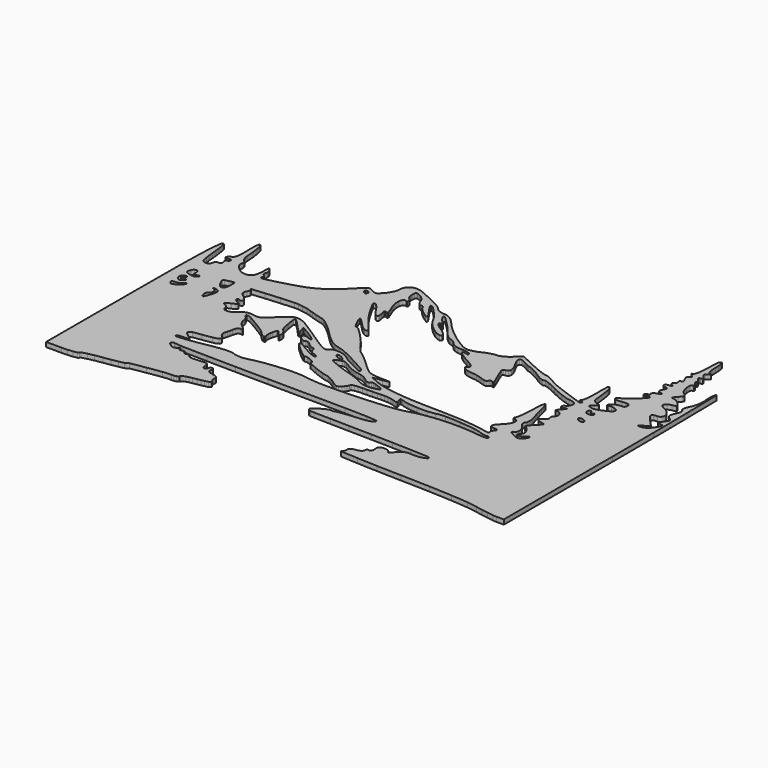
from build123d import *

# Parameters (mm, degrees)
F1_DEPTH = 3.175


# Not quite as in the source:
# - ends of sketch curves that miss each other by under 0.0002 mm in the source are joined


with BuildPart() as f1:
    # F0 (on Top) → F1 (new body)
    with BuildSketch(Plane.XY):
        with BuildLine():
            ThreePointArc((136.1546106763, 106.2652964117), (136.0578263341, 105.9058474976), (136.0076068165, 105.5369996552))
            ThreePointArc((136.0076068165, 105.5369996552), (135.9692871964, 104.9552365256), (135.9376510981, 104.3730716005))
            ThreePointArc((135.9376510981, 104.3730716005), (135.877045604, 103.1072283571), (135.8182378075, 101.841300329))
            ThreePointArc((135.8182378075, 101.841300329), (135.7507467659, 100.3377514915), (135.6857657927, 98.8340920952))
            ThreePointArc((135.6857657927, 98.8340920952), (135.6190340336, 97.2325909124), (135.5545194964, 95.6309988878))
            ThreePointArc((135.5545194964, 95.6309988878), (135.4619323702, 94.0261952793), (135.3115258719, 92.4257756303))
            ThreePointArc((135.3115258719, 92.4257756303), (135.1229682421, 91.1393543374), (134.8479637593, 89.8686039127))
            ThreePointArc((134.8479637593, 89.8686039127), (134.5810197829, 88.9631811201), (134.2428899921, 88.0818643691))
            ThreePointArc((134.2428899921, 88.0818643691), (133.9577029759, 87.7390624925), (133.5318894373, 87.6066800706))
            ThreePointArc((133.5318894373, 87.6066800706), (133.3013089072, 87.5654012055), (133.0961780229, 87.452301317))
            ThreePointArc((133.0961780229, 87.452301317), (132.9932475874, 87.2994752433), (132.9986083151, 87.1152915404))
            ThreePointArc((132.9986083151, 87.1152915404), (133.1387065215, 86.8328863427), (133.3421323889, 86.592061273))
            ThreePointArc((133.3421323889, 86.592061273), (133.7166250382, 86.2665055301), (134.1119890465, 85.9666401117))
            ThreePointArc((134.1119890465, 85.9666401117), (134.6429393341, 85.5675398211), (135.1498354606, 85.1383012897))
            ThreePointArc((135.1498354606, 85.1383012897), (135.3661134616, 84.8654092844), (135.4796990006, 84.536252161))
            ThreePointArc((135.4796990006, 84.536252161), (135.4509842396, 84.2590107261), (135.2853376336, 84.0348458786))
            ThreePointArc((135.2853376336, 84.0348458786), (134.9112753464, 83.7803948067), (134.5051684063, 83.5810323536))
            ThreePointArc((134.5051684063, 83.5810323536), (134.0877253763, 83.357167657), (133.7269885123, 83.0501751748))
            ThreePointArc((133.7269885123, 83.0501751748), (133.5010780971, 82.7139023508), (133.3984505089, 82.3220084737))
            ThreePointArc((133.3984505089, 82.3220084737), (133.4102112102, 81.8086601614), (133.5350286063, 81.3105777251))
            ThreePointArc((133.5350286063, 81.3105777251), (133.8324679678, 80.5880116296), (134.177796599, 79.8870696724))
            ThreePointArc((134.177796599, 79.8870696724), (134.5162185399, 79.2152319379), (134.8209500656, 78.5274572129))
            ThreePointArc((134.8209500656, 78.5274572129), (134.9466914957, 78.0990069656), (134.9787697775, 77.6536421823))
            ThreePointArc((134.9787697775, 77.6536421823), (134.9025321053, 77.3751256789), (134.7095329592, 77.1603261421))
            ThreePointArc((134.7095329592, 77.1603261421), (134.4077572859, 77.0127383461), (134.075678, 76.962))
            ThreePointArc((134.075678, 76.962), (133.786032802, 76.9345947435), (133.5066864431, 76.8532781187))
            ThreePointArc((133.5066864431, 76.8532781187), (133.3044976891, 76.7295975551), (133.1555317611, 76.545251297))
            ThreePointArc((133.1555317611, 76.545251297), (133.0770716363, 76.321598056), (133.0782244439, 76.0845831902))
            ThreePointArc((133.0782244439, 76.0845831902), (133.1559665272, 75.8041664896), (133.2849377373, 75.5433161484))
            ThreePointArc((133.2849377373, 75.5433161484), (133.4236296254, 75.2442392416), (133.487704414, 74.9208568419))
            ThreePointArc((133.487704414, 74.9208568419), (133.4792893246, 74.5714011953), (133.401381526, 74.2306373013))
            ThreePointArc((133.401381526, 74.2306373013), (133.2495258217, 73.8876195317), (133.0376193692, 73.5780734231))
            ThreePointArc((133.0376193692, 73.5780734231), (132.7647099375, 73.2985134436), (132.4501531896, 73.0668100349))
            ThreePointArc((132.4501531896, 73.0668100349), (132.0980188084, 72.8112929515), (131.787528817, 72.5065234816))
            ThreePointArc((131.787528817, 72.5065234816), (131.6443407877, 72.2462555102), (131.6241057565, 71.9498957575))
            ThreePointArc((131.6241057565, 71.9498957575), (131.7300721288, 71.6295758089), (131.937009965, 71.3630886919))
            ThreePointArc((131.937009965, 71.3630886919), (132.3570843274, 71.0119053057), (132.8062943541, 70.6988532593))
            ThreePointArc((132.8062943541, 70.6988532593), (133.3092100642, 70.3657457839), (133.7982428751, 70.0125720451))
            ThreePointArc((133.7982428751, 70.0125720451), (133.9064120821, 69.85041116), (133.8897787888, 69.6561964773))
            ThreePointArc((133.8897787888, 69.6561964773), (133.7524605442, 69.4904165732), (133.5495177242, 69.4186215518))
            ThreePointArc((133.5495177242, 69.4186215518), (132.8786708636, 69.381599599), (132.207000057, 69.3653360875))
            ThreePointArc((132.207000057, 69.3653360875), (131.693529434, 69.3325410929), (131.1867819409, 69.2434551141))
            ThreePointArc((131.1867819409, 69.2434551141), (130.7423930453, 69.1043928799), (130.3234276368, 68.9012001726))
            ThreePointArc((130.3234276368, 68.9012001726), (130.0103943601, 68.6782905535), (129.7440033369, 68.4013185416))
            ThreePointArc((129.7440033369, 68.4013185416), (129.5924726327, 68.126980599), (129.54, 67.818))
            ThreePointArc((129.54, 67.818), (129.586078691, 67.5137522476), (129.7201818483, 67.2367932546))
            ThreePointArc((129.7201818483, 67.2367932546), (129.9493772706, 66.9642945798), (130.2272731747, 66.7416749612))
            ThreePointArc((130.2272731747, 66.7416749612), (130.5926024118, 66.5438899228), (130.9850811445, 66.407711715))
            ThreePointArc((130.9850811445, 66.407711715), (131.4287501758, 66.3225384199), (131.8796194, 66.294))
            ThreePointArc((131.8796194, 66.294), (132.4263729059, 66.2574212951), (132.9633813281, 66.1483371424))
            ThreePointArc((132.9633813281, 66.1483371424), (133.2509368049, 65.9801574867), (133.415768116, 65.6906691262))
            ThreePointArc((133.415768116, 65.6906691262), (133.4550860432, 65.2732890195), (133.3597168136, 64.8650514964))
            ThreePointArc((133.3597168136, 64.8650514964), (133.0223810478, 64.1019295332), (132.647233384, 63.3566674874))
            ThreePointArc((132.647233384, 63.3566674874), (132.2769313234, 62.6027306022), (131.9600287022, 61.8248378774))
            ThreePointArc((131.9600287022, 61.8248378774), (131.8678470043, 61.3493625904), (131.9304478905, 60.8690943228))
            ThreePointArc((131.9304478905, 60.8690943228), (132.1352903447, 60.4831591111), (132.4730382703, 60.2059731037))
            ThreePointArc((132.4730382703, 60.2059731037), (133.0906045303, 59.9209918214), (133.7366144597, 59.708215766))
            ThreePointArc((133.7366144597, 59.708215766), (134.4398851068, 59.5056411898), (135.1347875125, 59.2759962248))
            ThreePointArc((135.1347875125, 59.2759962248), (135.2878109707, 59.1348928852), (135.2905053929, 58.9267569806))
            ThreePointArc((135.2905053929, 58.9267569806), (135.1327653444, 58.6969111367), (134.8955947141, 58.550415895))
            ThreePointArc((134.8955947141, 58.550415895), (133.9436548084, 58.2171736191), (132.9861459007, 57.9002877983))
            ThreePointArc((132.9861459007, 57.9002877983), (132.3521096202, 57.6670082208), (131.7396121179, 57.3819322011))
            ThreePointArc((131.7396121179, 57.3819322011), (131.2575791493, 57.0878732238), (130.8217404561, 56.7288874446))
            ThreePointArc((130.8217404561, 56.7288874446), (130.5548195268, 56.4155521231), (130.3595090394, 56.053226591))
            ThreePointArc((130.3595090394, 56.053226591), (130.3122258652, 55.7470358841), (130.4090865604, 55.4527466991))
            ThreePointArc((130.4090865604, 55.4527466991), (130.5311676955, 55.204554509), (130.6033906264, 54.9375574225))
            ThreePointArc((130.6033906264, 54.9375574225), (130.6022465182, 54.7112994769), (130.5245619672, 54.4987946658))
            ThreePointArc((130.5245619672, 54.4987946658), (130.3784301548, 54.3227065952), (130.1820576275, 54.2052348214))
            ThreePointArc((130.1820576275, 54.2052348214), (129.9107856233, 54.1280256079), (129.6299414, 54.102))
            ThreePointArc((129.6299414, 54.102), (129.3167864221, 54.0737499334), (129.0137610821, 53.9898381614))
            ThreePointArc((129.0137610821, 53.9898381614), (128.736597735, 53.8540886307), (128.4901054159, 53.6683808385))
            ThreePointArc((128.4901054159, 53.6683808385), (128.2909985409, 53.4461757723), (128.1397000369, 53.1890214598))
            ThreePointArc((128.1397000369, 53.1890214598), (128.047288767, 52.9141504411), (128.016, 52.6258536))
            ThreePointArc((128.016, 52.6258536), (128.0642564801, 52.3643478858), (128.2026693633, 52.1372888621))
            ThreePointArc((128.2026693633, 52.1372888621), (128.4232731315, 51.9534444099), (128.6875026464, 51.8409790635))
            ThreePointArc((128.6875026464, 51.8409790635), (129.0549838098, 51.7830062711), (129.4266642162, 51.7990396376))
            ThreePointArc((129.4266642162, 51.7990396376), (129.8707057739, 51.8884830825), (130.302001567, 52.0268921165))
            ThreePointArc((130.302001567, 52.0268921165), (130.7361143609, 52.1782853555), (131.1787334579, 52.3026319131))
            ThreePointArc((131.1787334579, 52.3026319131), (131.5448689193, 52.3714075289), (131.9164746403, 52.3977734899))
            ThreePointArc((131.9164746403, 52.3977734899), (132.1676461723, 52.3779175087), (132.4109080766, 52.3123075934))
            ThreePointArc((132.4109080766, 52.3123075934), (132.5393755297, 52.2126956072), (132.588, 52.0575794))
            ThreePointArc((132.588, 52.0575794), (132.4302267102, 51.2191838693), (131.9784916739, 50.4954885372))
            ThreePointArc((131.9784916739, 50.4954885372), (130.3891978995, 48.8175953901), (128.7526881254, 47.1857200947))
            ThreePointArc((128.7526881254, 47.1857200947), (127.0106651685, 45.5653908492), (125.2037478989, 44.0177609368))
            ThreePointArc((125.2037478989, 44.0177609368), (123.8011947114, 42.9795401235), (122.3010012363, 42.0882040571))
            ThreePointArc((122.3010012363, 42.0882040571), (120.8036344969, 41.233922886), (119.3657053193, 40.282995223))
            ThreePointArc((119.3657053193, 40.282995223), (118.993960134, 39.72907647), (119.0831048322, 39.0679577801))
            ThreePointArc((119.0831048322, 39.0679577801), (119.6173717028, 38.5157588574), (120.3604148756, 38.3201995501))
            ThreePointArc((120.3604148756, 38.3201995501), (122.2864064023, 38.3977814402), (124.2060019977, 38.5727530881))
            ThreePointArc((124.2060019977, 38.5727530881), (125.564765549, 38.7046361824), (126.9276350218, 38.7834984619))
            ThreePointArc((126.9276350218, 38.7834984619), (127.6981701336, 38.7397869434), (128.4465838007, 38.5513410382))
            ThreePointArc((128.4465838007, 38.5513410382), (128.909121907, 38.2824351382), (129.2431872909, 37.8645228272))
            ThreePointArc((129.2431872909, 37.8645228272), (129.4646757025, 37.2884863653), (129.54, 36.675949))
            ThreePointArc((129.54, 36.675949), (129.5039576679, 36.2007383086), (129.3966477689, 35.7364013226))
            ThreePointArc((129.3966477689, 35.7364013226), (129.2269080262, 35.3402654164), (128.9804197398, 34.9867412522))
            ThreePointArc((128.9804197398, 34.9867412522), (128.6971101847, 34.7280139709), (128.3604790066, 34.543938685))
            ThreePointArc((128.3604790066, 34.543938685), (128.0032022253, 34.4544479524), (127.6350017921, 34.4635693138))
            ThreePointArc((127.6350017921, 34.4635693138), (126.548111657, 34.5333189386), (125.4678216087, 34.3948747995))
            ThreePointArc((125.4678216087, 34.3948747995), (124.2126263008, 34.0348913029), (123.0055965143, 33.5367111286))
            ThreePointArc((123.0055965143, 33.5367111286), (121.9706315378, 32.9635940912), (121.0092398021, 32.2741450058))
            ThreePointArc((121.0092398021, 32.2741450058), (120.5571652457, 31.7009890971), (120.396, 30.989016))
            ThreePointArc((120.396, 30.989016), (120.4235379858, 30.7403825716), (120.5048170629, 30.5038014355))
            ThreePointArc((120.5048170629, 30.5038014355), (120.6276841876, 30.3325881754), (120.8032666059, 30.2160502161))
            ThreePointArc((120.8032666059, 30.2160502161), (121.0247760122, 30.1603422252), (121.2526166653, 30.1764374543))
            ThreePointArc((121.2526166653, 30.1764374543), (121.5264235324, 30.2641846009), (121.782454473, 30.3950189249))
            ThreePointArc((121.782454473, 30.3950189249), (122.5148399282, 30.7002895538), (123.3058976624, 30.761908692))
            ThreePointArc((123.3058976624, 30.761908692), (124.4173592826, 30.6057768822), (125.5028905829, 30.320565048))
            ThreePointArc((125.5028905829, 30.320565048), (126.4907533449, 29.930677501), (127.4244949526, 29.4246971051))
            ThreePointArc((127.4244949526, 29.4246971051), (127.8582009068, 28.9687365057), (128.016, 28.3595572))
            ThreePointArc((128.016, 28.3595572), (127.7462595657, 27.3192314332), (127.0050058769, 26.5410408576))
            ThreePointArc((127.0050058769, 26.5410408576), (125.0320778835, 25.4079209648), (122.9853913186, 24.4142015464))
            ThreePointArc((122.9853913186, 24.4142015464), (120.8097329546, 23.5454884195), (118.575173525, 22.8419989693))
            ThreePointArc((118.575173525, 22.8419989693), (117.1337543879, 22.6626032687), (115.7006141771, 22.8991900434))
            ThreePointArc((115.7006141771, 22.8991900434), (114.7495163619, 23.2163530426), (113.8080580116, 23.5610790158))
            ThreePointArc((113.8080580116, 23.5610790158), (113.5521376523, 23.7470214521), (113.424019411, 24.0362508715))
            ThreePointArc((113.424019411, 24.0362508715), (113.4573456204, 24.3524672546), (113.6429633216, 24.6106314062))
            ThreePointArc((113.6429633216, 24.6106314062), (114.4335236622, 25.242176866), (115.2417311971, 25.8509759099))
            ThreePointArc((115.2417311971, 25.8509759099), (116.0530753116, 26.461517055), (116.8473806031, 27.0940661827))
            ThreePointArc((116.8473806031, 27.0940661827), (117.0334837403, 27.3496711801), (117.0709597031, 27.6636222572))
            ThreePointArc((117.0709597031, 27.6636222572), (116.9489486458, 27.9495506635), (116.6984006368, 28.1335880815))
            ThreePointArc((116.6984006368, 28.1335880815), (115.7734634689, 28.4730444127), (114.8388840482, 28.7849743902))
            ThreePointArc((114.8388840482, 28.7849743902), (114.2299412478, 29.0120877951), (113.6465142369, 29.2984526133))
            ThreePointArc((113.6465142369, 29.2984526133), (113.1070817971, 29.635796743), (112.6063016944, 30.0282345625))
            ThreePointArc((112.6063016944, 30.0282345625), (112.2092609744, 30.4184357545), (111.8610203819, 30.8527482486))
            ThreePointArc((111.8610203819, 30.8527482486), (111.6605995236, 31.2296940161), (111.5621467398, 31.6450993388))
            ThreePointArc((111.5621467398, 31.6450993388), (110.9041596908, 37.4292607425), (110.1472498915, 43.2013102492))
            ThreePointArc((110.1472498915, 43.2013102492), (109.6108949095, 45.3687467535), (108.6399660857, 47.3794077002))
            ThreePointArc((108.6399660857, 47.3794077002), (107.940020907, 47.6610345513), (107.4633657459, 47.0762073865))
            ThreePointArc((107.4633657459, 47.0762073865), (107.3264782828, 42.7796862449), (107.33794468, 38.481000169))
            ThreePointArc((107.33794468, 38.481000169), (107.3498607646, 36.5874821362), (107.3101713047, 34.6943426933))
            ThreePointArc((107.3101713047, 34.6943426933), (107.2195000741, 32.9422899055), (107.068850292, 31.1943721968))
            ThreePointArc((107.068850292, 31.1943721968), (106.8970041584, 29.7509820247), (106.6808671001, 28.3135572185))
            ThreePointArc((106.6808671001, 28.3135572185), (106.4909399565, 27.651940466), (106.1552634787, 27.0509985024))
            ThreePointArc((106.1552634787, 27.0509985024), (105.8922853158, 26.6462379036), (105.6694602837, 26.21805813))
            ThreePointArc((105.6694602837, 26.21805813), (105.5958173077, 25.927721726), (105.6311127724, 25.6302781943))
            ThreePointArc((105.6311127724, 25.6302781943), (105.7652578038, 25.406049603), (105.9871647841, 25.2680995717))
            ThreePointArc((105.9871647841, 25.2680995717), (106.362402586, 25.1767146607), (106.7473862, 25.146))
            ThreePointArc((106.7473862, 25.146), (107.1002029429, 25.1329483991), (107.4510910755, 25.0938649407))
            ThreePointArc((107.4510910755, 25.0938649407), (107.690416808, 25.0324201998), (107.9120200434, 24.9231293434))
            ThreePointArc((107.9120200434, 24.9231293434), (108.01668347, 24.8157819177), (108.0609650763, 24.6725435225))
            ThreePointArc((108.0609650763, 24.6725435225), (108.0378434628, 24.5183249193), (107.9532712264, 24.3873073736))
            ThreePointArc((107.9532712264, 24.3873073736), (107.1260968805, 23.9263442832), (106.1801341517, 23.9694904046))
            ThreePointArc((106.1801341517, 23.9694904046), (100.9651706755, 25.737739547), (95.7657200347, 27.5510961735))
            ThreePointArc((95.7657200347, 27.5510961735), (90.8353642523, 29.3568259846), (85.9465929926, 31.2722851817))
            ThreePointArc((85.9465929926, 31.2722851817), (82.9558383129, 32.6324915411), (80.0905388969, 34.2402341139))
            ThreePointArc((80.0905388969, 34.2402341139), (79.0571559952, 34.8525780418), (78.0016692517, 35.425982768))
            ThreePointArc((78.0016692517, 35.425982768), (76.9458814353, 35.9480825657), (75.8702783685, 36.4280349896))
            ThreePointArc((75.8702783685, 36.4280349896), (74.930110244, 36.803668754), (73.9757962678, 37.141753782))
            ThreePointArc((73.9757962678, 37.141753782), (73.376889676, 37.2886446227), (72.7622116, 37.3380254))
            ThreePointArc((72.7622116, 37.3380254), (72.0461288224, 37.3973490273), (71.3495706237, 37.5737024024))
            ThreePointArc((71.3495706237, 37.5737024024), (69.7385259081, 38.1417982758), (68.1372473222, 38.7368657549))
            ThreePointArc((68.1372473222, 38.7368657549), (66.2287920541, 39.4870394566), (64.3362254159, 40.2764398117))
            ThreePointArc((64.3362254159, 40.2764398117), (62.2957129877, 41.1718984361), (60.2698834189, 42.100096632))
            Line((60.2698834189, 42.100096632), (50.0935752, 46.8621618))
            Line((50.0935752, 46.8621618), (45.9183994, 42.8620936))
            ThreePointArc((45.9183994, 42.8620936), (45.0121644888, 42.0595919188), (44.0458200441, 41.3305858515))
            ThreePointArc((44.0458200441, 41.3305858515), (42.9826946842, 40.6450941377), (41.8749821171, 40.0342690205))
            ThreePointArc((41.8749821171, 40.0342690205), (40.8246368377, 39.5479959143), (39.7420792863, 39.1384185314))
            ThreePointArc((39.7420792863, 39.1384185314), (38.8909211666, 38.9256397805), (38.0166118205, 38.8526192441))
            ThreePointArc((38.0166118205, 38.8526192441), (37.14320148, 38.8103066443), (36.2773461304, 38.6881151565))
            ThreePointArc((36.2773461304, 38.6881151565), (35.1841856218, 38.456935998), (34.1024233877, 38.1772329482))
            ThreePointArc((34.1024233877, 38.1772329482), (32.9775564787, 37.8326732973), (31.8688715584, 37.4391439626))
            ThreePointArc((31.8688715584, 37.4391439626), (30.8839939708, 37.031505982), (29.9248042018, 36.5666323819))
            ThreePointArc((29.9248042018, 36.5666323819), (28.9737390807, 36.1038940507), (27.9983439441, 35.6949244274))
            ThreePointArc((27.9983439441, 35.6949244274), (26.916577657, 35.303207448), (25.8188407843, 34.9587745794))
            ThreePointArc((25.8188407843, 34.9587745794), (24.7755902787, 34.6810270755), (23.7210595841, 34.4497681199))
            ThreePointArc((23.7210595841, 34.4497681199), (22.902874355, 34.3300328728), (22.0769434, 34.29))
            ThreePointArc((22.0769434, 34.29), (19.7470456182, 34.5868592428), (17.5660258354, 35.4584679803))
            ThreePointArc((17.5660258354, 35.4584679803), (13.8765734126, 37.625849264), (10.2963952395, 39.9693343977))
            ThreePointArc((10.2963952395, 39.9693343977), (6.4459178909, 42.7776909889), (2.7487381951, 45.7849997596))
            ThreePointArc((2.7487381951, 45.7849997596), (-0.4412414102, 48.7221846945), (-3.4182981909, 51.874986202))
            ThreePointArc((-3.4182981909, 51.874986202), (-4.9199157112, 53.5172312357), (-6.4825209745, 55.1015568026))
            ThreePointArc((-6.4825209745, 55.1015568026), (-7.7008807386, 56.1843945155), (-9.015158827, 57.1485579789))
            ThreePointArc((-9.015158827, 57.1485579789), (-10.133537645, 57.7917266206), (-11.3250938584, 58.2863319218))
            ThreePointArc((-11.3250938584, 58.2863319218), (-12.4760219855, 58.5764213281), (-13.6589262, 58.674))
            ThreePointArc((-13.6589262, 58.674), (-14.5522960105, 58.7190927137), (-15.4365949652, 58.8538370626))
            ThreePointArc((-15.4365949652, 58.8538370626), (-16.3585967303, 59.0830893313), (-17.2580542474, 59.3890637718))
            ThreePointArc((-17.2580542474, 59.3890637718), (-18.0730179036, 59.7470497227), (-18.8534459544, 60.1751291708))
            ThreePointArc((-18.8534459544, 60.1751291708), (-19.4330800045, 60.596621691), (-19.9349824824, 61.1082125833))
            ThreePointArc((-19.9349824824, 61.1082125833), (-21.4628041611, 62.6274455179), (-23.2511890469, 63.829101063))
            ThreePointArc((-23.2511890469, 63.829101063), (-27.2402506934, 65.9215797892), (-31.2826129874, 67.9091385908))
            ThreePointArc((-31.2826129874, 67.9091385908), (-35.3762453416, 69.7914909702), (-39.5171559332, 71.5674238037))
            ThreePointArc((-39.5171559332, 71.5674238037), (-41.5470231352, 72.1823582359), (-43.6577994, 72.39))
            ThreePointArc((-43.6577994, 72.39), (-45.0159606839, 72.261352582), (-46.325812574, 71.8799862783))
            ThreePointArc((-46.325812574, 71.8799862783), (-47.4705145108, 71.2727266991), (-48.455108221, 70.4302985429))
            ThreePointArc((-48.455108221, 70.4302985429), (-49.2574665677, 69.3684576557), (-49.8185832282, 68.1616326458))
            ThreePointArc((-49.8185832282, 68.1616326458), (-50.1728419756, 66.7564410752), (-50.292, 65.3121884))
            ThreePointArc((-50.292, 65.3121884), (-50.3540587338, 64.5023531368), (-50.5387857215, 63.7114293857))
            ThreePointArc((-50.5387857215, 63.7114293857), (-50.8988020714, 62.6902995432), (-51.325465817, 61.6951732046))
            ThreePointArc((-51.325465817, 61.6951732046), (-51.8616469844, 60.6391082438), (-52.4636981293, 59.6191582142))
            ThreePointArc((-52.4636981293, 59.6191582142), (-53.1038987179, 58.6860191563), (-53.8101836115, 57.8018438226))
            ThreePointArc((-53.8101836115, 57.8018438226), (-54.859126527, 56.6289370845), (-55.9525531925, 55.497385129))
            ThreePointArc((-55.9525531925, 55.497385129), (-56.5777605761, 55.0143075268), (-57.3032855425, 54.7014788531))
            ThreePointArc((-57.3032855425, 54.7014788531), (-57.9927469672, 54.6225862095), (-58.6697368063, 54.7751156362))
            ThreePointArc((-58.6697368063, 54.7751156362), (-59.7016185905, 55.2503471307), (-60.6897444701, 55.8109112473))
            ThreePointArc((-60.6897444701, 55.8109112473), (-61.6974651027, 56.3608474202), (-62.7626634966, 56.7889641118))
            ThreePointArc((-62.7626634966, 56.7889641118), (-63.5393276692, 56.9068133416), (-64.3099748746, 56.7545071496))
            ThreePointArc((-64.3099748746, 56.7545071496), (-65.2116195559, 56.2997012084), (-66.0059554068, 55.676130644))
            ThreePointArc((-66.0059554068, 55.676130644), (-67.5612052483, 54.1458828542), (-69.0775206326, 52.57704647))
            ThreePointArc((-69.0775206326, 52.57704647), (-73.1029047906, 48.5270797754), (-77.3374560644, 44.6963467451))
            ThreePointArc((-77.3374560644, 44.6963467451), (-80.950113618, 41.9073175477), (-84.8298501979, 39.5036493472))
            ThreePointArc((-84.8298501979, 39.5036493472), (-89.1893828189, 37.3603351246), (-93.7285444452, 35.6296349075))
            ThreePointArc((-93.7285444452, 35.6296349075), (-100.170724636, 33.6363437631), (-106.679998752, 31.8744550395))
            ThreePointArc((-106.679998752, 31.8744550395), (-109.9668031482, 31.0591673669), (-113.2589608177, 30.2657729718))
            ThreePointArc((-113.2589608177, 30.2657729718), (-114.5425209285, 30.014471266), (-115.8420084049, 29.8661047631))
            ThreePointArc((-115.8420084049, 29.8661047631), (-116.2967522502, 29.9553869778), (-116.6422934286, 30.2641970577))
            ThreePointArc((-116.6422934286, 30.2641970577), (-116.7729788265, 30.6991863385), (-116.6510606497, 31.1367082543))
            ThreePointArc((-116.6510606497, 31.1367082543), (-116.5102682382, 31.4328432562), (-116.4372805691, 31.7525143198))
            ThreePointArc((-116.4372805691, 31.7525143198), (-116.4321474779, 32.0912816786), (-116.4941350638, 32.4243679996))
            ThreePointArc((-116.4941350638, 32.4243679996), (-116.624268733, 32.7518302286), (-116.8137340668, 33.0489324198))
            ThreePointArc((-116.8137340668, 33.0489324198), (-117.0595526644, 33.312237131), (-117.3479889984, 33.5280178008))
            ThreePointArc((-117.3479889984, 33.5280178008), (-117.6364958642, 33.7435073287), (-117.8828615558, 34.0061387407))
            ThreePointArc((-117.8828615558, 34.0061387407), (-118.0729245927, 34.3019194451), (-118.2040680664, 34.6281288065))
            ThreePointArc((-118.2040680664, 34.6281288065), (-118.2670893675, 34.9591105612), (-118.2632936594, 35.2960183191))
            ThreePointArc((-118.2632936594, 35.2960183191), (-118.1917750455, 35.6133456994), (-118.0523649212, 35.907241868))
            ThreePointArc((-118.0523649212, 35.907241868), (-117.8937011692, 36.2577950018), (-117.8293571155, 36.6371632678))
            ThreePointArc((-117.8293571155, 36.6371632678), (-117.8358280437, 37.1641529555), (-117.8966977853, 37.6876552189))
            ThreePointArc((-117.8966977853, 37.6876552189), (-118.026193524, 38.2830955904), (-118.2106179846, 38.8638764261))
            ThreePointArc((-118.2106179846, 38.8638764261), (-118.4524459336, 39.4399376835), (-118.7431809012, 39.9929293506))
            ThreePointArc((-118.7431809012, 39.9929293506), (-119.1478051941, 40.6434946075), (-119.5895888309, 41.2694209807))
            ThreePointArc((-119.5895888309, 41.2694209807), (-119.8051020284, 41.3770316963), (-120.0204180538, 41.2690368705))
            ThreePointArc((-120.0204180538, 41.2690368705), (-120.2094139009, 40.9156186531), (-120.2849156423, 40.5220166063))
            ThreePointArc((-120.2849156423, 40.5220166063), (-120.3270632679, 39.1830762927), (-120.3496776958, 37.8436635138))
            ThreePointArc((-120.3496776958, 37.8436635138), (-120.4413197127, 35.4913548699), (-120.6708078773, 33.1484738738))
            ThreePointArc((-120.6708078773, 33.1484738738), (-121.015690477, 31.6720764625), (-121.6539665491, 30.2968291376))
            ThreePointArc((-121.6539665491, 30.2968291376), (-122.4131435278, 29.38350615), (-123.4165683452, 28.7481779987))
            ThreePointArc((-123.4165683452, 28.7481779987), (-124.7275743835, 28.3339976038), (-126.0953028, 28.194))
            ThreePointArc((-126.0953028, 28.194), (-127.7596557184, 28.3983115931), (-129.3251749798, 28.9991138121))
            ThreePointArc((-129.3251749798, 28.9991138121), (-131.0390434838, 30.0714825249), (-132.5852045422, 31.3740561016))
            ThreePointArc((-132.5852045422, 31.3740561016), (-133.8169425379, 32.7658818173), (-134.8245344196, 34.3276491932))
            ThreePointArc((-134.8245344196, 34.3276491932), (-135.1805781203, 35.5597091464), (-134.9882976898, 36.8276877135))
            ThreePointArc((-134.9882976898, 36.8276877135), (-134.874437597, 37.2384171579), (-134.8410147707, 37.6633230362))
            ThreePointArc((-134.8410147707, 37.6633230362), (-134.8849453518, 38.1155263111), (-134.9998146027, 38.5550977168))
            ThreePointArc((-134.9998146027, 38.5550977168), (-135.1848396232, 38.977176548), (-135.4332852041, 39.3653244306))
            ThreePointArc((-135.4332852041, 39.3653244306), (-135.7303446061, 39.6935668339), (-136.0803088641, 39.9646968235))
            ThreePointArc((-136.0803088641, 39.9646968235), (-136.490256568, 40.304813205), (-136.8063709531, 40.7335396464))
            ThreePointArc((-136.8063709531, 40.7335396464), (-137.1600284078, 41.4251283854), (-137.4556196303, 42.1434553944))
            ThreePointArc((-137.4556196303, 42.1434553944), (-137.7323822718, 43.0040246698), (-137.9428980952, 43.8831494183))
            ThreePointArc((-137.9428980952, 43.8831494183), (-138.0919566505, 44.7974504641), (-138.17602148, 45.7200002178))
            ThreePointArc((-138.17602148, 45.7200002178), (-138.3454155571, 48.2257153493), (-138.5748813752, 50.7266448233))
            ThreePointArc((-138.5748813752, 50.7266448233), (-138.8375160501, 52.8577384684), (-139.1814411245, 54.9772318309))
            ThreePointArc((-139.1814411245, 54.9772318309), (-139.5156577451, 56.6372961456), (-139.9116929434, 58.2837077813))
            ThreePointArc((-139.9116929434, 58.2837077813), (-140.2210884225, 59.0418926277), (-140.7184462941, 59.6924305059))
            ThreePointArc((-140.7184462941, 59.6924305059), (-141.1088949395, 59.8025052632), (-141.4066644401, 59.5269870278))
            ThreePointArc((-141.4066644401, 59.5269870278), (-141.6750951676, 58.5113255321), (-141.8301833551, 57.4723017531))
            ThreePointArc((-141.8301833551, 57.4723017531), (-141.9693958317, 55.4647281726), (-142.0127900739, 53.4528014157))
            ThreePointArc((-142.0127900739, 53.4528014157), (-141.9860081676, 50.1315731978), (-141.9207021016, 46.8108790599))
            ThreePointArc((-141.9207021016, 46.8108790599), (-141.9150382413, 45.3093962039), (-141.9745492209, 43.8090820838))
            ThreePointArc((-141.9745492209, 43.8090820838), (-142.1009329571, 42.7187084447), (-142.344187716, 41.6483283215))
            ThreePointArc((-142.344187716, 41.6483283215), (-142.6254282641, 40.8975747158), (-143.0239746347, 40.2019540931))
            ThreePointArc((-143.0239746347, 40.2019540931), (-143.4663471089, 39.7290427651), (-144.0292085586, 39.4088552548))
            ThreePointArc((-144.0292085586, 39.4088552548), (-144.4763192889, 39.2088426311), (-144.8991960024, 38.9616856039))
            ThreePointArc((-144.8991960024, 38.9616856039), (-145.2851294111, 38.6742305579), (-145.6357810194, 38.3446568044))
            ThreePointArc((-145.6357810194, 38.3446568044), (-145.9083688328, 38.0180218975), (-146.1372129805, 37.6593803407))
            ThreePointArc((-146.1372129805, 37.6593803407), (-146.2616381704, 37.3462186345), (-146.304, 37.0119148))
            ThreePointArc((-146.304, 37.0119148), (-146.2559430297, 36.7418660472), (-146.1176728334, 36.5049754521))
            ThreePointArc((-146.1176728334, 36.5049754521), (-145.8982672698, 36.313044478), (-145.6324980584, 36.1932803693))
            ThreePointArc((-145.6324980584, 36.1932803693), (-145.2655266123, 36.1291278426), (-144.8931837987, 36.1411115128))
            ThreePointArc((-144.8931837987, 36.1411115128), (-144.4490972909, 36.2277449194), (-144.0179999279, 36.365129012))
            ThreePointArc((-144.0179999279, 36.365129012), (-143.5867057739, 36.5035423175), (-143.1426644612, 36.592987465))
            ThreePointArc((-143.1426644612, 36.592987465), (-142.7709928618, 36.6090196425), (-142.4035196978, 36.5510528008))
            ThreePointArc((-142.4035196978, 36.5510528008), (-142.1392916899, 36.4385669315), (-141.9186740947, 36.2547323042))
            ThreePointArc((-141.9186740947, 36.2547323042), (-141.7802564801, 36.0276775142), (-141.732, 35.7661718))
            ThreePointArc((-141.732, 35.7661718), (-141.7604485607, 35.4789161308), (-141.8446889818, 35.2028206916))
            ThreePointArc((-141.8446889818, 35.2028206916), (-141.9817074643, 34.9475178404), (-142.1656408682, 34.7236408682))
            ThreePointArc((-142.1656408682, 34.7236408682), (-142.3895081005, 34.5397139875), (-142.6448073182, 34.4027178396))
            ThreePointArc((-142.6448073182, 34.4027178396), (-142.9209046357, 34.3184508601), (-143.2081718, 34.29))
            ThreePointArc((-143.2081718, 34.29), (-143.4696854251, 34.2417658972), (-143.6967491599, 34.1033447425))
            ThreePointArc((-143.6967491599, 34.1033447425), (-143.8805605254, 33.8827187928), (-143.9930209365, 33.6184973536))
            ThreePointArc((-143.9930209365, 33.6184973536), (-144.0509937289, 33.2510161902), (-144.0349603624, 32.8793357838))
            ThreePointArc((-144.0349603624, 32.8793357838), (-143.9455180637, 32.4352986293), (-143.8071111437, 32.0040069289))
            ThreePointArc((-143.8071111437, 32.0040069289), (-143.6664691228, 31.5307081761), (-143.6006277996, 31.0413653663))
            ThreePointArc((-143.6006277996, 31.0413653663), (-143.6418280263, 30.6629481161), (-143.8031734589, 30.3181811785))
            ThreePointArc((-143.8031734589, 30.3181811785), (-144.0673588942, 30.0440552129), (-144.4059824961, 29.8700619844))
            ThreePointArc((-144.4059824961, 29.8700619844), (-144.8865641345, 29.7562436409), (-145.3789574, 29.718))
            ThreePointArc((-145.3789574, 29.718), (-145.8544260206, 29.6741529684), (-146.3138569891, 29.5440908426))
            ThreePointArc((-146.3138569891, 29.5440908426), (-146.735128382, 29.3334722851), (-147.1085894955, 29.0464934459))
            ThreePointArc((-147.1085894955, 29.0464934459), (-147.4113920255, 28.7017732009), (-147.6404350809, 28.304205496))
            ThreePointArc((-147.6404350809, 28.304205496), (-147.7805806601, 27.8780734052), (-147.828, 27.432))
            ThreePointArc((-147.828, 27.432), (-147.9849727571, 26.6390367347), (-148.432213684, 25.9656818951))
            ThreePointArc((-148.432213684, 25.9656818951), (-149.1300186958, 25.4612337976), (-149.9526837563, 25.2070300607))
            ThreePointArc((-149.9526837563, 25.2070300607), (-150.8952110685, 25.2116021263), (-151.799011242, 25.4790433968))
            ThreePointArc((-151.799011242, 25.4790433968), (-152.5789360059, 25.9857509341), (-153.1785316172, 26.6967485379))
            ThreePointArc((-153.1785316172, 26.6967485379), (-153.4273625763, 27.189822164), (-153.5878944784, 27.718280715))
            ThreePointArc((-153.5878944784, 27.718280715), (-153.8304654495, 28.9239867737), (-154.048450058, 30.1343795781))
            ThreePointArc((-154.048450058, 30.1343795781), (-154.2777961105, 31.5920357819), (-154.472311981, 33.0547469364))
            ThreePointArc((-154.472311981, 33.0547469364), (-154.6482569257, 34.6367150997), (-154.7940664919, 36.2217449728))
            ThreePointArc((-154.7940664919, 36.2217449728), (-154.9441024158, 37.8891825592), (-155.1192069871, 39.5541742737))
            ThreePointArc((-155.1192069871, 39.5541742737), (-155.3241139353, 41.2649622842), (-155.552600364, 42.9727609544))
            ThreePointArc((-155.552600364, 42.9727609544), (-155.777562894, 44.4940436491), (-156.023531158, 46.0120715627))
            ThreePointArc((-156.023531158, 46.0120715627), (-156.2161682383, 47.0138557806), (-156.453523497, 48.0059963967))
            ThreePointArc((-156.453523497, 48.0059963967), (-157.2531708199, 48.5918206677), (-157.9916576902, 47.9305620145))
            ThreePointArc((-157.9916576902, 47.9305620145), (-158.688933033, 42.6195853082), (-159.0806076134, 37.277370254))
            ThreePointArc((-159.0806076134, 37.277370254), (-159.510328698, 25.1773747548), (-159.7220156678, 13.0716018565))
            ThreePointArc((-159.7220156678, 13.0716018565), (-159.8660340939, -8.5135094991), (-159.9321687417, -30.0989999976))
            Line((-159.9321687417, -30.0989999976), (-160.02, -99.822))
            Line((-160.02, -99.822), (-149.479, -99.822))
            ThreePointArc((-149.479, -99.822), (-147.4400540376, -99.7943434538), (-145.40260565, -99.7114689333))
            ThreePointArc((-145.40260565, -99.7114689333), (-143.6403017242, -99.5791373388), (-141.8850090374, -99.3737702744))
            ThreePointArc((-141.8850090374, -99.3737702744), (-140.4922982289, -99.1582972434), (-139.1073382649, -98.8976096333))
            ThreePointArc((-139.1073382649, -98.8976096333), (-138.6878039938, -98.6876605897), (-138.4293612487, -98.2961301171))
            ThreePointArc((-138.4293612487, -98.2961301171), (-138.1618280589, -97.8717530574), (-137.728145673, -97.6195711944))
            ThreePointArc((-137.728145673, -97.6195711944), (-136.001445693, -97.1311354909), (-134.2651110751, -96.6781408996))
            ThreePointArc((-134.2651110751, -96.6781408996), (-132.124031035, -96.1784486694), (-129.9683229389, -95.7461995343))
            ThreePointArc((-129.9683229389, -95.7461995343), (-127.4720480383, -95.3127922577), (-124.9673904653, -94.9307977404))
            ThreePointArc((-124.9673904653, -94.9307977404), (-122.4556956444, -94.5600815894), (-119.9481984161, -94.1619630684))
            ThreePointArc((-119.9481984161, -94.1619630684), (-117.7684547165, -93.7852137277), (-115.5952212162, -93.3725639579))
            ThreePointArc((-115.5952212162, -93.3725639579), (-113.7659732266, -93.0019921496), (-111.9397309663, -92.6168809667))
            ThreePointArc((-111.9397309663, -92.6168809667), (-111.5626339755, -92.4691236885), (-111.2519981301, -92.2092406154))
            ThreePointArc((-111.2519981301, -92.2092406154), (-110.5013976136, -91.5921039521), (-109.5878434306, -91.2609264871))
            ThreePointArc((-109.5878434306, -91.2609264871), (-104.4752122961, -90.3595002287), (-99.357102279, -89.4897209209))
            ThreePointArc((-99.357102279, -89.4897209209), (-94.4967114429, -88.7179768484), (-89.6249138036, -88.0218620741))
            ThreePointArc((-89.6249138036, -88.0218620741), (-86.7148843512, -87.7280520011), (-83.7917044, -87.6299746))
            ThreePointArc((-83.7917044, -87.6299746), (-82.9197949052, -87.6044724202), (-82.0508662177, -87.5280560317))
            ThreePointArc((-82.0508662177, -87.5280560317), (-81.3097121525, -87.4064867842), (-80.582721873, -87.2178763429))
            ThreePointArc((-80.582721873, -87.2178763429), (-80.0572891307, -87.0219646863), (-79.5577768063, -86.7671139249))
            ThreePointArc((-79.5577768063, -86.7671139249), (-79.3309406582, -86.5383706433), (-79.248, -86.2270818))
            ThreePointArc((-79.248, -86.2270818), (-79.1696110702, -85.8926293327), (-78.950772173, -85.6278410884))
            ThreePointArc((-78.950772173, -85.6278410884), (-78.4430486252, -85.2779759372), (-77.904981432, -84.9768555359))
            ThreePointArc((-77.904981432, -84.9768555359), (-77.1780798865, -84.6494224696), (-76.4271466953, -84.3816624615))
            ThreePointArc((-76.4271466953, -84.3816624615), (-75.5577098612, -84.1369826952), (-74.6760008561, -83.941077368))
            ThreePointArc((-74.6760008561, -83.941077368), (-73.6301652704, -83.7390141741), (-72.5843587891, -83.5368003963))
            ThreePointArc((-72.5843587891, -83.5368003963), (-71.3220495349, -83.292569479), (-70.0597550587, -83.0482621982))
            ThreePointArc((-70.0597550587, -83.0482621982), (-68.7902933261, -82.8024560452), (-67.5208477494, -82.5565664731))
            ThreePointArc((-67.5208477494, -82.5565664731), (-66.4510964921, -82.3492787497), (-65.3813771458, -82.1418264032))
            ThreePointArc((-65.3813771458, -82.1418264032), (-64.346566026, -81.916621449), (-63.3230146944, -81.6447882671))
            ThreePointArc((-63.3230146944, -81.6447882671), (-62.7322767007, -81.410666099), (-62.1964697888, -81.0690558334))
            ThreePointArc((-62.1964697888, -81.0690558334), (-61.9634299267, -80.775205078), (-61.8906007031, -80.4073076809))
            ThreePointArc((-61.8906007031, -80.4073076809), (-61.9831533245, -80.0082852305), (-62.2142961642, -79.6701159642))
            ThreePointArc((-62.2142961642, -79.6701159642), (-62.5125806463, -79.3227076957), (-62.7548917369, -78.9341833852))
            ThreePointArc((-62.7548917369, -78.9341833852), (-62.955451823, -78.4853980592), (-63.0994878356, -78.0154130065))
            ThreePointArc((-63.0994878356, -78.0154130065), (-63.1824101332, -77.5416258096), (-63.2054201604, -77.0611868611))
            ThreePointArc((-63.2054201604, -77.0611868611), (-63.1613728862, -76.6341988179), (-63.0433571859, -76.2214890194))
            ThreePointArc((-63.0433571859, -76.2214890194), (-62.9766429279, -75.7975980569), (-63.088813341, -75.3834095103))
            ThreePointArc((-63.088813341, -75.3834095103), (-63.3823645483, -74.9471212984), (-63.7694599535, -74.5912028393))
            ThreePointArc((-63.7694599535, -74.5912028393), (-64.4007074949, -74.2018361449), (-65.0819886131, -73.9086925937))
            ThreePointArc((-65.0819886131, -73.9086925937), (-66.0032299499, -73.6245106999), (-66.9416263436, -73.4034727181))
            ThreePointArc((-66.9416263436, -73.4034727181), (-68.0172390042, -73.1562007301), (-69.0769770309, -72.8479131584))
            ThreePointArc((-69.0769770309, -72.8479131584), (-69.7239317349, -72.564328828), (-70.3004692222, -72.1561932547))
            ThreePointArc((-70.3004692222, -72.1561932547), (-70.6235831363, -71.7557791423), (-70.7904634368, -71.2690730775))
            ThreePointArc((-70.7904634368, -71.2690730775), (-70.8049107174, -70.7008837458), (-70.6721188813, -70.148238173))
            ThreePointArc((-70.6721188813, -70.148238173), (-70.5349519489, -69.7093321381), (-70.45451928, -69.2565798812))
            ThreePointArc((-70.45451928, -69.2565798812), (-70.4536610705, -68.8750342757), (-70.5361412214, -68.5025083499))
            ThreePointArc((-70.5361412214, -68.5025083499), (-70.6788387906, -68.2272815416), (-70.8966847787, -68.0066987148))
            ThreePointArc((-70.8966847787, -68.0066987148), (-71.1655691038, -67.8664123361), (-71.4649574, -67.818))
            ThreePointArc((-71.4649574, -67.818), (-71.7921595589, -67.8471631925), (-72.1090465199, -67.933733387))
            ThreePointArc((-72.1090465199, -67.933733387), (-72.3985154028, -68.0736799286), (-72.6564277369, -68.2656670996))
            ThreePointArc((-72.6564277369, -68.2656670996), (-72.8642596204, -68.4948338921), (-73.0226421888, -68.7605919452))
            ThreePointArc((-73.0226421888, -68.7605919452), (-73.1192665728, -69.0441892113), (-73.152, -69.342))
            ThreePointArc((-73.152, -69.342), (-73.1813714862, -69.6385684944), (-73.2683447792, -69.9236144597))
            ThreePointArc((-73.2683447792, -69.9236144597), (-73.4097885787, -70.1871914407), (-73.599682637, -70.4183173628))
            ThreePointArc((-73.599682637, -70.4183173628), (-73.8308118812, -70.6082052577), (-74.0943923043, -70.7496389902))
            ThreePointArc((-74.0943923043, -70.7496389902), (-74.3794362962, -70.836604072), (-74.676, -70.8659746))
            ThreePointArc((-74.676, -70.8659746), (-74.9877810718, -70.807996964), (-75.2578430356, -70.6417491833))
            ThreePointArc((-75.2578430356, -70.6417491833), (-75.5339357779, -70.3426634786), (-75.7523207748, -69.9991720178))
            ThreePointArc((-75.7523207748, -69.9991720178), (-75.9532045212, -69.5334246525), (-76.0875549805, -69.0443172668))
            ThreePointArc((-76.0875549805, -69.0443172668), (-76.1718161913, -68.4825024526), (-76.2, -67.9151042))
            ThreePointArc((-76.2, -67.9151042), (-76.279025898, -67.1358190785), (-76.5128859908, -66.3882631608))
            ThreePointArc((-76.5128859908, -66.3882631608), (-76.8623036178, -65.8933273163), (-77.3834659158, -65.5843858416))
            ThreePointArc((-77.3834659158, -65.5843858416), (-78.2634255872, -65.3765714575), (-79.1666193059, -65.3346224605))
            ThreePointArc((-79.1666193059, -65.3346224605), (-81.1139137014, -65.4479435032), (-83.0579986181, -65.6070971416))
            ThreePointArc((-83.0579986181, -65.6070971416), (-84.5120795995, -65.7176371608), (-85.969145188, -65.7770424587))
            ThreePointArc((-85.969145188, -65.7770424587), (-87.0438525265, -65.7559868846), (-88.112827312, -65.6431417585))
            ThreePointArc((-88.112827312, -65.6431417585), (-88.8103814477, -65.4914331192), (-89.4818127039, -65.2489938941))
            ThreePointArc((-89.4818127039, -65.2489938941), (-89.7978199634, -64.9816225408), (-89.916, -64.5849102))
            ThreePointArc((-89.916, -64.5849102), (-89.9634469495, -64.2893893136), (-90.1010184902, -64.0235738166))
            ThreePointArc((-90.1010184902, -64.0235738166), (-90.3172077669, -63.8082505961), (-90.5875071577, -63.6666961486))
            ThreePointArc((-90.5875071577, -63.6666961486), (-90.9528350557, -63.5844946448), (-91.327298551, -63.5844698571))
            ThreePointArc((-91.327298551, -63.5844698571), (-91.7714571806, -63.6627803818), (-92.2019957052, -63.7971149919))
            ThreePointArc((-92.2019957052, -63.7971149919), (-92.6326409097, -63.9320166959), (-93.0768007991, -64.0118660008))
            ThreePointArc((-93.0768007991, -64.0118660008), (-93.4508558674, -64.0140293412), (-93.8164966812, -63.9351168437))
            ThreePointArc((-93.8164966812, -63.9351168437), (-94.08598634, -63.7975818412), (-94.3027216853, -63.5864727264))
            ThreePointArc((-94.3027216853, -63.5864727264), (-94.4404398779, -63.3259355435), (-94.488, -63.0351038))
            ThreePointArc((-94.488, -63.0351038), (-94.5355601221, -62.7442720565), (-94.6732854876, -62.4837403081))
            ThreePointArc((-94.6732854876, -62.4837403081), (-94.8900234513, -62.2726187379), (-95.1595236807, -62.1350756418))
            ThreePointArc((-95.1595236807, -62.1350756418), (-95.5251575664, -62.0561768654), (-95.8992000037, -62.0583600512))
            ThreePointArc((-95.8992000037, -62.0583600512), (-96.3433546715, -62.1382152193), (-96.7739967912, -62.2731121619))
            ThreePointArc((-96.7739967912, -62.2731121619), (-97.2045450238, -62.4074843653), (-97.6487002592, -62.4859262774))
            ThreePointArc((-97.6487002592, -62.4859262774), (-98.0231346666, -62.486101813), (-98.3885025165, -62.4041999409))
            ThreePointArc((-98.3885025165, -62.4041999409), (-98.6587421237, -62.2630100667), (-98.874964029, -62.0480366449))
            ThreePointArc((-98.874964029, -62.0480366449), (-99.0125418206, -61.7826721422), (-99.06, -61.487558))
            ThreePointArc((-99.06, -61.487558), (-99.0900847857, -61.1587957771), (-99.1793397981, -60.84095425))
            ThreePointArc((-99.1793397981, -60.84095425), (-99.311152805, -60.6697753759), (-99.5153970162, -60.5993301664))
            ThreePointArc((-99.5153970162, -60.5993301664), (-99.811340817, -60.6331878848), (-100.0829019533, -60.7555912899))
            ThreePointArc((-100.0829019533, -60.7555912899), (-100.5354835314, -61.0697750191), (-100.9693350531, -61.4093562523))
            ThreePointArc((-100.9693350531, -61.4093562523), (-101.4596621409, -61.750163448), (-102.0007406383, -62.0027584048))
            ThreePointArc((-102.0007406383, -62.0027584048), (-102.5316667012, -62.1330677428), (-103.07825356, -62.1434762985))
            ThreePointArc((-103.07825356, -62.1434762985), (-103.6872684653, -62.0305370876), (-104.2655208258, -61.8085510852))
            ThreePointArc((-104.2655208258, -61.8085510852), (-104.9669655594, -61.4240341208), (-105.6325151041, -60.9802750492))
            ThreePointArc((-105.6325151041, -60.9802750492), (-106.4770211968, -60.2630272725), (-107.2086669584, -59.4309642504))
            ThreePointArc((-107.2086669584, -59.4309642504), (-107.3597139807, -58.8707353784), (-107.0778985951, -58.3635263773))
            ThreePointArc((-107.0778985951, -58.3635263773), (-106.3238352421, -57.9515255826), (-105.4733734024, -57.8287756867))
            ThreePointArc((-105.4733734024, -57.8287756867), (-103.7862621921, -57.9360740861), (-102.1079988107, -58.139271276))
            ThreePointArc((-102.1079988107, -58.139271276), (-100.6768122252, -58.3067716063), (-99.2377742511, -58.3810689557))
            ThreePointArc((-99.2377742511, -58.3810689557), (-90.8217366567, -58.5379218112), (-82.4055503395, -58.686581124))
            ThreePointArc((-82.4055503395, -58.686581124), (-72.6308013042, -58.8416011733), (-62.8556781292, -58.9708946528))
            ThreePointArc((-62.8556781292, -58.9708946528), (-51.6209383495, -59.0949218322), (-40.3860000265, -59.1994275465))
            ThreePointArc((-40.3860000265, -59.1994275465), (-13.8292614298, -59.4315074955), (12.7273302669, -59.6798283778))
            ThreePointArc((12.7273302669, -59.6798283778), (20.3437516045, -59.8066735987), (27.957652634, -60.0400725199))
            ThreePointArc((27.957652634, -60.0400725199), (31.4169996192, -60.257003218), (34.8611935119, -60.6464491922))
            ThreePointArc((34.8611935119, -60.6464491922), (35.5319918526, -61.2026159111), (35.3327072837, -62.0508910837))
            ThreePointArc((35.3327072837, -62.0508910837), (34.8043504491, -62.4796722942), (34.1990656282, -62.7905464998))
            ThreePointArc((34.1990656282, -62.7905464998), (33.1730910815, -63.1574748924), (32.1285663013, -63.4676833799))
            ThreePointArc((32.1285663013, -63.4676833799), (30.8878461617, -63.7643864378), (29.6331150915, -63.9947533056))
            ThreePointArc((29.6331150915, -63.9947533056), (28.333401488, -64.165325665), (27.0268949571, -64.2720506399))
            ThreePointArc((27.0268949571, -64.2720506399), (24.6729559145, -64.4297155314), (22.3225874633, -64.6338120532))
            ThreePointArc((22.3225874633, -64.6338120532), (19.7794937423, -64.899885139), (17.2408334315, -65.2053754061))
            ThreePointArc((17.2408334315, -65.2053754061), (14.952104616, -65.5129214025), (12.6672630113, -65.8481266193))
            ThreePointArc((12.6672630113, -65.8481266193), (11.6541423493, -66.057064822), (10.6679946206, -66.3694490413))
            ThreePointArc((10.6679946206, -66.3694490413), (10.4826417567, -66.4276472041), (10.2920792117, -66.4654444699))
            ThreePointArc((10.2920792117, -66.4654444699), (10.0369031642, -66.4956245903), (9.7805747541, -66.5135566003))
            ThreePointArc((9.7805747541, -66.5135566003), (9.5043323794, -66.5197789943), (9.2281004514, -66.5131290354))
            ThreePointArc((9.2281004514, -66.5131290354), (8.9717558948, -66.4935310626), (8.7169767336, -66.4591160878))
            ThreePointArc((8.7169767336, -66.4591160878), (7.6460958204, -66.4448442554), (6.6187694566, -66.7474883896))
            ThreePointArc((6.6187694566, -66.7474883896), (4.6965180409, -67.6980514281), (2.8196983607, -68.735436954))
            ThreePointArc((2.8196983607, -68.735436954), (0.9893996903, -69.851138127), (-0.7957030735, -71.0378095317))
            ThreePointArc((-0.7957030735, -71.0378095317), (-1.3309154405, -71.6439175684), (-1.524, -72.429116))
            ThreePointArc((-1.524, -72.429116), (-1.4718441106, -72.7336994598), (-1.3213194484, -73.0035765555))
            ThreePointArc((-1.3213194484, -73.0035765555), (-1.0534340945, -73.2812557221), (-0.7405690031, -73.5070523148))
            ThreePointArc((-0.7405690031, -73.5070523148), (-0.3217186178, -73.7170804986), (0.1227255348, -73.8654635403))
            ThreePointArc((0.1227255348, -73.8654635403), (0.6289087856, -73.9667421827), (1.1430004035, -74.0135063891))
            ThreePointArc((1.1430004035, -74.0135063891), (2.1392008282, -74.0462470723), (3.1356553115, -74.0700367655))
            ThreePointArc((3.1356553115, -74.0700367655), (8.7889638962, -74.1792661607), (14.4422876968, -74.2877051331))
            ThreePointArc((14.4422876968, -74.2877051331), (21.0140828553, -74.4120488197), (27.5859241377, -74.5339302988))
            ThreePointArc((27.5859241377, -74.5339302988), (35.1289453929, -74.6714560225), (42.6720004971, -74.8071123681))
            ThreePointArc((42.6720004971, -74.8071123681), (50.2020149101, -74.9575021411), (57.7313295031, -75.1395866909))
            ThreePointArc((57.7313295031, -75.1395866909), (64.2612532127, -75.3322905235), (70.7898004426, -75.5670461043))
            ThreePointArc((70.7898004426, -75.5670461043), (76.4123070727, -75.7938093962), (82.034278223, -76.0334816431))
            ThreePointArc((82.034278223, -76.0334816431), (82.9434898636, -76.1507854638), (83.8199952729, -76.4194169689))
            ThreePointArc((83.8199952729, -76.4194169689), (84.1946884055, -76.8843953355), (83.9939295861, -77.44679878))
            ThreePointArc((83.9939295861, -77.44679878), (83.0303371338, -78.1148242477), (81.9431435346, -78.5538953965))
            ThreePointArc((81.9431435346, -78.5538953965), (79.8543243688, -79.0362865553), (77.7301986982, -79.3260409848))
            ThreePointArc((77.7301986982, -79.3260409848), (75.6489292562, -79.4094942833), (73.5696772105, -79.285570148))
            ThreePointArc((73.5696772105, -79.285570148), (72.5120897956, -79.2346156899), (71.4561931374, -79.3131671357))
            ThreePointArc((71.4561931374, -79.3131671357), (70.4908937491, -79.5197838331), (69.5675985762, -79.8690971601))
            ThreePointArc((69.5675985762, -79.8690971601), (68.6327634662, -80.3854411379), (67.7759628209, -81.0229517905))
            ThreePointArc((67.7759628209, -81.0229517905), (66.825592302, -81.9004218682), (65.945184363, -82.8480712044))
            ThreePointArc((65.945184363, -82.8480712044), (65.2957035416, -83.5703825933), (64.6150339624, -84.2633817455))
            ThreePointArc((64.6150339624, -84.2633817455), (64.0830948598, -84.7265845862), (63.502798699, -85.1275488861))
            ThreePointArc((63.502798699, -85.1275488861), (63.1688918537, -85.267968379), (62.8083577243, -85.3029841172))
            ThreePointArc((62.8083577243, -85.3029841172), (62.5794263764, -85.1971943977), (62.4858797855, -84.9629999733))
            ThreePointArc((62.4858797855, -84.9629999733), (62.4094744456, -84.5707398642), (62.1921451637, -84.2353747057))
            ThreePointArc((62.1921451637, -84.2353747057), (61.7958788039, -83.8895655557), (61.3457300864, -83.6175758221))
            ThreePointArc((61.3457300864, -83.6175758221), (60.7324750191, -83.3658445792), (60.0910902706, -83.1982901197))
            ThreePointArc((60.0910902706, -83.1982901197), (59.3524549987, -83.0931251469), (58.607198, -83.0579746))
            ThreePointArc((58.607198, -83.0579746), (57.8502954171, -83.0917245144), (57.0994004582, -83.1927063807))
            ThreePointArc((57.0994004582, -83.1927063807), (56.4880094506, -83.3517692844), (55.9078902522, -83.6018922046))
            ThreePointArc((55.9078902522, -83.6018922046), (55.5087105667, -83.8704353162), (55.1769292798, -84.2188317773))
            ThreePointArc((55.1769292798, -84.2188317773), (55.0037228728, -84.5712114083), (54.9777582918, -84.963001079))
            ThreePointArc((54.9777582918, -84.963001079), (55.1070830934, -86.2370112934), (55.1649823291, -87.5162589324))
            ThreePointArc((55.1649823291, -87.5162589324), (55.1066356836, -88.387199959), (54.9032267689, -89.236062033))
            ThreePointArc((54.9032267689, -89.236062033), (54.6518998429, -89.67118964), (54.2482808493, -89.9705132576))
            ThreePointArc((54.2482808493, -89.9705132576), (53.7872742281, -90.057658278), (53.3400081297, -89.9159868453))
            ThreePointArc((53.3400081297, -89.9159868453), (53.0619259843, -89.7907165105), (52.7609560687, -89.7413282581))
            ThreePointArc((52.7609560687, -89.7413282581), (52.495440483, -89.7829102124), (52.2636722736, -89.9189686825))
            ThreePointArc((52.2636722736, -89.9189686825), (52.0578123574, -90.1590957664), (51.9282918516, -90.4476469573))
            ThreePointArc((51.9282918516, -90.4476469573), (51.8442063189, -90.8443140959), (51.816, -91.2488142))
            ThreePointArc((51.816, -91.2488142), (51.7384326782, -91.7461555042), (51.5130987134, -92.1962551226))
            ThreePointArc((51.5130987134, -92.1962551226), (51.1211744423, -92.6509662827), (50.652277347, -93.025803896))
            ThreePointArc((50.652277347, -93.025803896), (50.0057174204, -93.387816627), (49.3141834869, -93.654040292))
            ThreePointArc((49.3141834869, -93.654040292), (48.4775723765, -93.8682291923), (47.6249998873, -94.0057546203))
            ThreePointArc((47.6249998873, -94.0057546203), (46.7458671534, -94.1418188529), (45.8800137892, -94.3459916093))
            ThreePointArc((45.8800137892, -94.3459916093), (45.2434137062, -94.5830277002), (44.6566596, -94.925319178))
            ThreePointArc((44.6566596, -94.925319178), (44.2786728606, -95.2726220811), (44.0019861294, -95.7049861173))
            ThreePointArc((44.0019861294, -95.7049861173), (43.872335503, -96.1608998275), (43.8954591043, -96.6343216798))
            ThreePointArc((43.8954591043, -96.6343216798), (43.9558022037, -97.0813422489), (43.9463508202, -97.5323177335))
            ThreePointArc((43.9463508202, -97.5323177335), (43.8683220782, -98.0007040435), (43.7288127952, -98.4545890889))
            ThreePointArc((43.7288127952, -98.4545890889), (43.5354007132, -98.8726339593), (43.2866269684, -99.2602962186))
            ThreePointArc((43.2866269684, -99.2602962186), (43.0097788308, -99.5673569843), (42.6801730268, -99.8169360588))
            ThreePointArc((42.6801730268, -99.8169360588), (42.5751804896, -100.0771057342), (42.7920915393, -100.2550382421))
            ThreePointArc((42.7920915393, -100.2550382421), (48.5896243665, -100.5573086792), (54.3878767889, -100.8454465542))
            ThreePointArc((54.3878767889, -100.8454465542), (61.2805237094, -101.1515038578), (68.1754286665, -101.4015793439))
            ThreePointArc((68.1754286665, -101.4015793439), (76.5325527277, -101.6515120768), (84.8907370543, -101.8630400392))
            ThreePointArc((84.8907370543, -101.8630400392), (94.9740310394, -102.1249550503), (105.0555942628, -102.446670331))
            ThreePointArc((105.0555942628, -102.446670331), (112.8283413128, -102.7673183498), (120.5963801358, -103.1868218878))
            ThreePointArc((120.5963801358, -103.1868218878), (126.4563998882, -103.585376237), (132.3096906421, -104.0728849311))
            ThreePointArc((132.3096906421, -104.0728849311), (135.8938770019, -104.5078335446), (139.4454399986, -105.1574280095))
            ThreePointArc((139.4454399986, -105.1574280095), (141.6654618417, -105.6133754653), (143.8928305758, -106.0319598926))
            ThreePointArc((143.8928305758, -106.0319598926), (146.160659794, -106.4196740797), (148.4344270608, -106.7708925093))
            ThreePointArc((148.4344270608, -106.7708925093), (150.4469201591, -107.0487998637), (152.4636019219, -107.2944739691))
            ThreePointArc((152.4636019219, -107.2944739691), (153.7629324541, -107.4050922662), (155.0664412, -107.442))
            Line((155.0664412, -107.442), (160.02, -107.442))
            Line((160.02, -107.442), (159.9128882, -14.097))
            ThreePointArc((159.9128882, -14.097), (159.8708387685, 3.6967045018), (159.7855244624, 21.4902541511))
            ThreePointArc((159.7855244624, 21.4902541511), (159.6656761158, 36.2117310228), (159.4830135358, 50.9325625264))
            ThreePointArc((159.4830135358, 50.9325625264), (159.2936875739, 63.5215979852), (159.0918874378, 76.1104396568))
            ThreePointArc((159.0918874378, 76.1104396568), (158.8826308922, 76.3570663773), (158.5998777361, 76.2000032687))
            ThreePointArc((158.5998777361, 76.2000032687), (158.3475979275, 75.434757879), (158.1860165314, 74.6453678702))
            ThreePointArc((158.1860165314, 74.6453678702), (158.0499350667, 73.5301111799), (157.9634914094, 72.4099134678))
            ThreePointArc((157.9634914094, 72.4099134678), (157.9224212166, 71.1730018364), (157.9348941161, 69.935471175))
            ThreePointArc((157.9348941161, 69.935471175), (158.0016763913, 68.7542073966), (158.12680724, 67.5776934448))
            ThreePointArc((158.12680724, 67.5776934448), (158.2476738547, 66.2556628091), (158.2637539138, 64.9282162842))
            ThreePointArc((158.2637539138, 64.9282162842), (158.1778662337, 63.5393842674), (157.9968837908, 62.1597192325))
            ThreePointArc((157.9968837908, 62.1597192325), (157.7221160249, 60.7984352902), (157.3544104705, 59.4592621981))
            ThreePointArc((157.3544104705, 59.4592621981), (156.9113259194, 58.216406696), (156.3701076924, 57.0130374668))
            ThreePointArc((156.3701076924, 57.0130374668), (155.8361264543, 55.8816036486), (155.3519520774, 54.7279771339))
            ThreePointArc((155.3519520774, 54.7279771339), (155.0732738472, 53.8800764985), (154.8946550242, 53.0056098632))
            ThreePointArc((154.8946550242, 53.0056098632), (154.8649161291, 52.3906303113), (154.9520475077, 51.7811277112))
            ThreePointArc((154.9520475077, 51.7811277112), (155.152917888, 51.3456348327), (155.5042843354, 51.0192240595))
            ThreePointArc((155.5042843354, 51.0192240595), (155.8626995004, 50.7093619621), (156.1060095058, 50.302819244))
            ThreePointArc((156.1060095058, 50.302819244), (156.2501434276, 49.7834004341), (156.27822539, 49.2450881433))
            ThreePointArc((156.27822539, 49.2450881433), (156.1845456111, 48.4998207875), (155.9909140337, 47.7740763389))
            ThreePointArc((155.9909140337, 47.7740763389), (155.6225727625, 46.7752830478), (155.2052833474, 45.7959295543))
            ThreePointArc((155.2052833474, 45.7959295543), (154.7002275314, 44.6183634998), (154.2482621121, 43.4194183913))
            ThreePointArc((154.2482621121, 43.4194183913), (154.085319519, 42.7171557736), (154.0797854736, 41.996259148))
            ThreePointArc((154.0797854736, 41.996259148), (154.2343967112, 41.4032309407), (154.5600647462, 40.8840668245))
            ThreePointArc((154.5600647462, 40.8840668245), (155.1622723655, 40.2623838539), (155.8308980197, 39.7127634539))
            ThreePointArc((155.8308980197, 39.7127634539), (156.5321070012, 39.1558352393), (157.1867588368, 38.5448574172))
            ThreePointArc((157.1867588368, 38.5448574172), (157.4761975439, 38.1184752783), (157.5931819557, 37.6165871799))
            ThreePointArc((157.5931819557, 37.6165871799), (157.5371043655, 37.0444682905), (157.3219142566, 36.5114055575))
            ThreePointArc((157.3219142566, 36.5114055575), (156.7142683749, 35.5153025868), (156.0651656342, 34.5457042976))
            ThreePointArc((156.0651656342, 34.5457042976), (155.3936728322, 33.5663313834), (154.7419075561, 32.5737206149))
            ThreePointArc((154.7419075561, 32.5737206149), (154.5708084931, 32.1945008745), (154.5170829524, 31.7819530754))
            ThreePointArc((154.5170829524, 31.7819530754), (154.6200190151, 31.5076748873), (154.8729178152, 31.3598010698))
            ThreePointArc((154.8729178152, 31.3598010698), (155.4954872608, 31.2715362352), (156.1235892, 31.2420254))
            ThreePointArc((156.1235892, 31.2420254), (156.9748545184, 31.1842508194), (157.8105073245, 31.0119866841))
            ThreePointArc((157.8105073245, 31.0119866841), (158.1989358123, 30.7461540172), (158.3436791124, 30.298288352))
            ThreePointArc((158.3436791124, 30.298288352), (158.2400510956, 29.5944920354), (157.959426876, 28.9407993469))
            ThreePointArc((157.959426876, 28.9407993469), (157.0144051798, 27.3867802326), (156.0347266021, 25.8543727359))
            ThreePointArc((156.0347266021, 25.8543727359), (155.4786311268, 25.0980270162), (154.8443624007, 24.4059269374))
            ThreePointArc((154.8443624007, 24.4059269374), (154.1239286641, 23.7676488099), (153.3433119312, 23.2045660097))
            ThreePointArc((153.3433119312, 23.2045660097), (152.5716627907, 22.7611776056), (151.7572029688, 22.4024423673))
            ThreePointArc((151.7572029688, 22.4024423673), (151.0503329892, 22.2090657902), (150.3197141971, 22.1520015224))
            ThreePointArc((150.3197141971, 22.1520015224), (149.2463069922, 22.1765369689), (148.1732881835, 22.2144222435))
            ThreePointArc((148.1732881835, 22.2144222435), (148.0166792679, 22.2916479829), (147.9685706282, 22.4595172268))
            ThreePointArc((147.9685706282, 22.4595172268), (148.0491561014, 22.6697970176), (148.2142536917, 22.8229485848))
            ThreePointArc((148.2142536917, 22.8229485848), (149.4042248917, 23.4983201368), (150.59851819, 24.1660188277))
            Line((150.59851819, 24.1660188277), (154.1310354, 26.126059))
            Line((154.1310354, 26.126059), (149.656038, 30.9165498))
            ThreePointArc((149.656038, 30.9165498), (148.1780813021, 32.5569117151), (146.7601506048, 34.2494297432))
            ThreePointArc((146.7601506048, 34.2494297432), (146.2963885509, 35.0756877453), (146.1307819215, 36.0086146794))
            ThreePointArc((146.1307819215, 36.0086146794), (146.3531793385, 36.6593978905), (146.9331826127, 37.0289615592))
            ThreePointArc((146.9331826127, 37.0289615592), (148.260686112, 37.260504699), (149.606, 37.3380254))
            ThreePointArc((149.606, 37.3380254), (150.8540988688, 37.6578625612), (151.7945550855, 38.5385377003))
            ThreePointArc((151.7945550855, 38.5385377003), (152.2611483664, 39.8151309693), (152.1478329404, 41.1695912826))
            ThreePointArc((152.1478329404, 41.1695912826), (151.3579272134, 42.9171797206), (150.1628707556, 44.4171335823))
            ThreePointArc((150.1628707556, 44.4171335823), (148.5614284603, 45.6892362612), (146.7342752427, 46.6081344081))
            ThreePointArc((146.7342752427, 46.6081344081), (145.4807498144, 47.2214467387), (144.3600891283, 48.0530683542))
            ThreePointArc((144.3600891283, 48.0530683542), (143.81995543, 48.8615068487), (143.7368429364, 49.8302287484))
            ThreePointArc((143.7368429364, 49.8302287484), (144.1309377801, 50.7660069409), (144.9028037305, 51.4257138536))
            ThreePointArc((144.9028037305, 51.4257138536), (146.2604365532, 51.9875869775), (147.6917790057, 52.3194334196))
            ThreePointArc((147.6917790057, 52.3194334196), (148.7473505425, 52.4920565435), (149.7966247376, 52.6995495216))
            ThreePointArc((149.7966247376, 52.6995495216), (150.1001854927, 52.8634719847), (150.2683196538, 53.164717068))
            ThreePointArc((150.2683196538, 53.164717068), (150.2671365847, 53.5380504743), (150.1010032166, 53.8723906181))
            ThreePointArc((150.1010032166, 53.8723906181), (149.3007566214, 54.8196182679), (148.4792040356, 55.7484269463))
            ThreePointArc((148.4792040356, 55.7484269463), (147.9098082219, 56.3309297644), (147.2973054754, 56.8679237254))
            ThreePointArc((147.2973054754, 56.8679237254), (146.6348465642, 57.3660995927), (145.9378095284, 57.8146186402))
            ThreePointArc((145.9378095284, 57.8146186402), (145.2861855673, 58.1676866254), (144.6091922033, 58.4692686158))
            ThreePointArc((144.6091922033, 58.4692686158), (144.0871504956, 58.622350901), (143.5455854, 58.6739999999))
            ThreePointArc((143.5455854, 58.6739999999), (143.0273060591, 58.7115073535), (142.5198115057, 58.8231659877))
            ThreePointArc((142.5198115057, 58.8231659877), (142.2959279077, 58.9930450526), (142.2398522684, 59.2684354489))
            ThreePointArc((142.2398522684, 59.2684354489), (142.3683400813, 59.6972980571), (142.603965223, 60.0779733292))
            ThreePointArc((142.603965223, 60.0779733292), (143.3115801723, 60.9210457929), (144.0399372881, 61.7462645222))
            ThreePointArc((144.0399372881, 61.7462645222), (144.8962473725, 62.7217266344), (145.7226538018, 63.7226491939))
            ThreePointArc((145.7226538018, 63.7226491939), (145.9711686783, 64.171779832), (146.0559840329, 64.6780266555))
            ThreePointArc((146.0559840329, 64.6780266555), (145.9556462371, 65.1421437797), (145.6753674994, 65.5254409469))
            ThreePointArc((145.6753674994, 65.5254409469), (144.8647370776, 66.2158468069), (144.0210027465, 66.8653805852))
            ThreePointArc((144.0210027465, 66.8653805852), (142.9738631546, 67.864755175), (142.2205818315, 69.1008072783))
            ThreePointArc((142.2205818315, 69.1008072783), (141.5643157172, 70.8663054305), (141.1267839884, 72.6983078652))
            ThreePointArc((141.1267839884, 72.6983078652), (140.966088947, 74.2895081431), (141.0388045101, 75.8871486871))
            ThreePointArc((141.0388045101, 75.8871486871), (141.4398507845, 76.6545237209), (142.249271, 76.9620254))
            ThreePointArc((142.249271, 76.9620254), (142.4517426852, 77.0169531076), (142.5986958674, 77.1666748448))
            ThreePointArc((142.5986958674, 77.1666748448), (142.6759390381, 77.3938028987), (142.6665519738, 77.6335274119))
            ThreePointArc((142.6665519738, 77.6335274119), (142.5463790776, 78.0141304182), (142.3647599352, 78.369537979))
            ThreePointArc((142.3647599352, 78.369537979), (142.0634225217, 78.8196043135), (141.7319945335, 79.2479954632))
            ThreePointArc((141.7319945335, 79.2479954632), (141.3948883044, 79.6781194238), (141.0823370059, 80.1264034774))
            ThreePointArc((141.0823370059, 80.1264034774), (140.8800689805, 80.4828795506), (140.7255564633, 80.8625022211))
            ThreePointArc((140.7255564633, 80.8625022211), (140.6835136448, 81.0962912218), (140.7095112739, 81.3324032375))
            ThreePointArc((140.7095112739, 81.3324032375), (140.8052976149, 81.4777317398), (140.97, 81.5340254))
            ThreePointArc((140.97, 81.5340254), (141.1347023851, 81.5902936602), (141.2304926382, 81.7356211498))
            ThreePointArc((141.2304926382, 81.7356211498), (141.2564863552, 81.9717341782), (141.2144416582, 82.2055225528))
            ThreePointArc((141.2144416582, 82.2055225528), (141.0599310195, 82.5851458494), (140.857662128, 82.9416213541))
            ThreePointArc((140.857662128, 82.9416213541), (140.5451175068, 83.3898981189), (140.2080097843, 83.8200081202))
            ThreePointArc((140.2080097843, 83.8200081202), (139.7302206196, 84.4159235336), (139.2728762325, 85.0276702995))
            ThreePointArc((139.2728762325, 85.0276702995), (139.1240398662, 85.3215444365), (139.0727724, 85.6469458))
            ThreePointArc((139.0727724, 85.6469458), (139.1484492339, 85.8680503224), (139.3436905939, 85.9964682364))
            ThreePointArc((139.3436905939, 85.9964682364), (139.7723866343, 86.0785297582), (140.208, 86.1060254))
            ThreePointArc((140.208, 86.1060254), (140.6233144433, 86.1378259127), (141.0289304476, 86.2325604507))
            ThreePointArc((141.0289304476, 86.2325604507), (141.2241892261, 86.3755850613), (141.2925050155, 86.6077770488))
            ThreePointArc((141.2925050155, 86.6077770488), (141.2269542757, 86.9572873742), (141.0640145619, 87.2733651582))
            ThreePointArc((141.0640145619, 87.2733651582), (140.5988524191, 87.8992763614), (140.1116226295, 88.5081671713))
            ThreePointArc((140.1116226295, 88.5081671713), (139.6059971775, 89.1575902693), (139.141864793, 89.8372882029))
            ThreePointArc((139.141864793, 89.8372882029), (138.9568275223, 90.2593625951), (138.9092053001, 90.7177518469))
            ThreePointArc((138.9092053001, 90.7177518469), (139.0087777103, 91.1252102767), (139.2512350481, 91.4674804635))
            ThreePointArc((139.2512350481, 91.4674804635), (139.7577130672, 91.9078038449), (140.3060002478, 92.294825862))
            ThreePointArc((140.3060002478, 92.294825862), (140.7876419393, 92.6125442466), (141.2568752801, 92.9483178866))
            ThreePointArc((141.2568752801, 92.9483178866), (141.4225399373, 93.1270201637), (141.5132591035, 93.3531780152))
            ThreePointArc((141.5132591035, 93.3531780152), (141.4811066719, 93.5202850741), (141.3409951343, 93.6168687231))
            ThreePointArc((141.3409951343, 93.6168687231), (140.967171015, 93.6788223804), (140.5889996723, 93.7026560574))
            ThreePointArc((140.5889996723, 93.7026560574), (140.1235080971, 93.8251424974), (139.7704756602, 94.1523329034))
            ThreePointArc((139.7704756602, 94.1523329034), (139.4201550389, 94.791720702), (139.1721253105, 95.4773013086))
            ThreePointArc((139.1721253105, 95.4773013086), (138.9336584016, 96.5349279623), (138.798318036, 97.6106246329))
            ThreePointArc((138.798318036, 97.6106246329), (138.7125911347, 99.0962139643), (138.684, 100.584))
            ThreePointArc((138.684, 100.584), (138.6610829275, 101.8992484735), (138.5923595321, 103.2129001907))
            ThreePointArc((138.5923595321, 103.2129001907), (138.4830532706, 104.3241796837), (138.3109359221, 105.4274772596))
            ThreePointArc((138.3109359221, 105.4274772596), (138.1335186207, 106.2562227416), (137.9103211226, 107.0738285526))
            ThreePointArc((137.9103211226, 107.0738285526), (137.7229925591, 107.3399263851), (137.414, 107.4420254))
            ThreePointArc((137.414, 107.4420254), (137.1559986489, 107.4049009145), (136.9189035505, 107.2966098547))
            ThreePointArc((136.9189035505, 107.2966098547), (136.6790551717, 107.1096698138), (136.4769794188, 106.8824233645))
            ThreePointArc((136.4769794188, 106.8824233645), (136.291911855, 106.5863349805), (136.1546106763, 106.2652964117))
        make_face()
        with BuildLine():
            ThreePointArc((-144.5915489955, -2.1001567798), (-145.1078207057, -2.5746237165), (-145.6532486165, -3.0152638723))
            ThreePointArc((-145.6532486165, -3.0152638723), (-146.8043681308, -3.8470043206), (-147.9909198005, -4.6273652967))
            ThreePointArc((-147.9909198005, -4.6273652967), (-148.7133014395, -4.97882196), (-149.4938127677, -5.1689672034))
            ThreePointArc((-149.4938127677, -5.1689672034), (-150.0881817656, -5.1358510709), (-150.6290033495, -4.8870771001))
            ThreePointArc((-150.6290033495, -4.8870771001), (-151.1873071587, -4.398943833), (-151.6379871736, -3.8099920727))
            ThreePointArc((-151.6379871736, -3.8099920727), (-151.7431725881, -3.5313229349), (-151.7358963511, -3.2335515547))
            ThreePointArc((-151.7358963511, -3.2335515547), (-151.6178288739, -2.953453938), (-151.4078560484, -2.7336674706))
            ThreePointArc((-151.4078560484, -2.7336674706), (-151.0388466595, -2.5227519766), (-150.6334066596, -2.3951843156))
            ThreePointArc((-150.6334066596, -2.3951843156), (-150.0853424122, -2.3133694206), (-149.5318828, -2.286))
            ThreePointArc((-149.5318828, -2.286), (-148.9087486768, -2.2558172552), (-148.2914487117, -2.16555161))
            ThreePointArc((-148.2914487117, -2.16555161), (-147.6794070298, -2.0153962209), (-147.0841401328, -1.8085194986))
            ThreePointArc((-147.0841401328, -1.8085194986), (-146.5705459864, -1.5715936757), (-146.0836082344, -1.2838369024))
            ThreePointArc((-146.0836082344, -1.2838369024), (-145.7476153502, -1.0050489509), (-145.4793260895, -0.6606106847))
            ThreePointArc((-145.4793260895, -0.6606106847), (-145.2721275003, -0.3681890681), (-145.0298581488, -0.104090918))
            ThreePointArc((-145.0298581488, -0.104090918), (-144.7869714215, 0.0877423508), (-144.511629061, 0.2290963845))
            ThreePointArc((-144.511629061, 0.2290963845), (-144.2647450719, 0.2920275786), (-144.0099711223, 0.2905944862))
            ThreePointArc((-144.0099711223, 0.2905944862), (-143.7859453143, 0.2222137627), (-143.595634189, 0.0856634102))
            ThreePointArc((-143.595634189, 0.0856634102), (-143.4645227872, -0.1460071561), (-143.4713454793, -0.4121136951))
            ThreePointArc((-143.4713454793, -0.4121136951), (-143.6262344651, -0.8132841305), (-143.8374299338, -1.1878827729))
            ThreePointArc((-143.8374299338, -1.1878827729), (-144.190531679, -1.6638239499), (-144.5915489955, -2.1001567798))
        make_face(mode=Mode.SUBTRACT)
        with BuildLine():
            ThreePointArc((-126.3269219689, 4.5892032812), (-125.940498176, 4.3932823038), (-125.5706202616, 4.1676748894))
            ThreePointArc((-125.5706202616, 4.1676748894), (-125.1717919866, 3.8041563007), (-124.9002143129, 3.3378366773))
            ThreePointArc((-124.9002143129, 3.3378366773), (-124.7284963728, 2.7344702878), (-124.6775378381, 2.109215781))
            ThreePointArc((-124.6775378381, 2.109215781), (-124.7450923819, 1.2183116312), (-124.9170596351, 0.3415569076))
            ThreePointArc((-124.9170596351, 0.3415569076), (-125.272659706, -0.9348698226), (-125.676567775, -2.1968428016))
            ThreePointArc((-125.676567775, -2.1968428016), (-126.1941172663, -3.6740792194), (-126.7359086318, -5.1425980721))
            ThreePointArc((-126.7359086318, -5.1425980721), (-126.9848448575, -5.6024695667), (-127.3469663144, -5.9797158872))
            ThreePointArc((-127.3469663144, -5.9797158872), (-127.6522622916, -6.0573455612), (-127.9129875384, -5.8805633279))
            ThreePointArc((-127.9129875384, -5.8805633279), (-128.2834372328, -5.2119966773), (-128.5901671208, -4.5119036463))
            ThreePointArc((-128.5901671208, -4.5119036463), (-128.7851617093, -3.9201866274), (-128.9223811693, -3.3124661302))
            ThreePointArc((-128.9223811693, -3.3124661302), (-128.972801203, -2.7864938234), (-128.94049949, -2.2590991962))
            ThreePointArc((-128.94049949, -2.2590991962), (-128.8386741201, -1.8525926126), (-128.6537166288, -1.4765535391))
            ThreePointArc((-128.6537166288, -1.4765535391), (-128.415851763, -1.2131165123), (-128.1032261357, -1.045049993))
            ThreePointArc((-128.1032261357, -1.045049993), (-127.4242266009, -0.6687483656), (-126.926472463, -0.073021932))
            ThreePointArc((-126.926472463, -0.073021932), (-126.6187886096, 0.7199472403), (-126.5449385822, 1.5673067274))
            ThreePointArc((-126.5449385822, 1.5673067274), (-126.7102560112, 2.4482306586), (-127.0978114032, 3.256409607))
            ThreePointArc((-127.0978114032, 3.256409607), (-127.6654038455, 3.8902801119), (-128.3970022712, 4.3246999713))
            ThreePointArc((-128.3970022712, 4.3246999713), (-128.7264786606, 4.4681274948), (-129.047705839, 4.6291846745))
            ThreePointArc((-129.047705839, 4.6291846745), (-129.193590221, 4.741929178), (-129.2947392897, 4.8960778563))
            ThreePointArc((-129.2947392897, 4.8960778563), (-129.296031462, 5.0126619929), (-129.212745436, 5.0942469266))
            ThreePointArc((-129.212745436, 5.0942469266), (-128.9990796258, 5.1590717319), (-128.7779994828, 5.1903548733))
            ThreePointArc((-128.7779994828, 5.1903548733), (-128.4243450814, 5.1909350429), (-128.0733285413, 5.1478140201))
            ThreePointArc((-128.0733285413, 5.1478140201), (-127.6368673826, 5.0523539217), (-127.2071865432, 4.9299407415))
            ThreePointArc((-127.2071865432, 4.9299407415), (-126.761881406, 4.7729359888), (-126.3269219689, 4.5892032812))
        make_face(mode=Mode.SUBTRACT)
        with BuildLine():
            ThreePointArc((-75.234216767, 17.6850760169), (-73.8259950496, 17.3170988337), (-72.4409524083, 16.8697147766))
            ThreePointArc((-72.4409524083, 16.8697147766), (-71.113106148, 16.4095696869), (-69.7787227891, 15.9687409256))
            ThreePointArc((-69.7787227891, 15.9687409256), (-68.3223111243, 15.5083466419), (-66.8607752773, 15.0644870845))
            ThreePointArc((-66.8607752773, 15.0644870845), (-65.4937677411, 14.6662916999), (-64.122297909, 14.2837484659))
            ThreePointArc((-64.122297909, 14.2837484659), (-63.1028324497, 14.0207389998), (-62.0764847599, 13.7860167824))
            ThreePointArc((-62.0764847599, 13.7860167824), (-60.929804364, 13.4286784193), (-59.8668274023, 12.8695310073))
            ThreePointArc((-59.8668274023, 12.8695310073), (-58.1454337122, 11.7043469895), (-56.4712963979, 10.4722294225))
            ThreePointArc((-56.4712963979, 10.4722294225), (-54.5298431943, 8.9220560134), (-52.6507235543, 7.296882872))
            ThreePointArc((-52.6507235543, 7.296882872), (-50.7140128375, 5.4963721122), (-48.8369434138, 3.6337671778))
            ThreePointArc((-48.8369434138, 3.6337671778), (-46.5267537709, 1.329909035), (-44.1539596994, -0.9094180047))
            ThreePointArc((-44.1539596994, -0.9094180047), (-42.3307930663, -2.4733702313), (-40.4065047109, -3.9110765303))
            ThreePointArc((-40.4065047109, -3.9110765303), (-38.7541345691, -4.9551941198), (-37.0155772927, -5.8484622634))
            ThreePointArc((-37.0155772927, -5.8484622634), (-35.2948495965, -6.5315029323), (-33.5122271045, -7.0312048452))
            ThreePointArc((-33.5122271045, -7.0312048452), (-30.4504541709, -7.8965642467), (-27.5008178013, -9.0894350091))
            ThreePointArc((-27.5008178013, -9.0894350091), (-22.8416942357, -11.3542068739), (-18.2465029408, -13.7460349558))
            ThreePointArc((-18.2465029408, -13.7460349558), (-13.5607998824, -16.3085948536), (-8.9104392981, -18.934746776))
            ThreePointArc((-8.9104392981, -18.934746776), (-8.042067965, -19.7763923157), (-7.6809085069, -20.9305143623))
            ThreePointArc((-7.6809085069, -20.9305143623), (-7.8904125118, -21.3574894402), (-8.3639323733, -21.4019198285))
            ThreePointArc((-8.3639323733, -21.4019198285), (-11.1387335664, -20.1468465621), (-13.8936705107, -18.8487506218))
            ThreePointArc((-13.8936705107, -18.8487506218), (-16.6393557412, -17.4770244238), (-19.3420449546, -16.0224139917))
            ThreePointArc((-19.3420449546, -16.0224139917), (-21.1533670667, -14.9050277983), (-22.8599979861, -13.6334729305))
            ThreePointArc((-22.8599979861, -13.6334729305), (-24.5119787908, -12.4912454144), (-26.3234149161, -11.6238219857))
            ThreePointArc((-26.3234149161, -11.6238219857), (-28.3740028038, -10.9836049133), (-30.4901343146, -10.6137683734))
            ThreePointArc((-30.4901343146, -10.6137683734), (-32.3423682106, -10.5490724999), (-34.1841842227, -10.755626672))
            ThreePointArc((-34.1841842227, -10.755626672), (-35.3396869788, -11.2494501998), (-36.1768417527, -12.1865882595))
            ThreePointArc((-36.1768417527, -12.1865882595), (-36.7733616347, -12.787711622), (-37.5946161417, -12.9944090489))
            ThreePointArc((-37.5946161417, -12.9944090489), (-38.7943936772, -12.8426232723), (-39.9392829805, -12.4530962167))
            ThreePointArc((-39.9392829805, -12.4530962167), (-42.0093199387, -11.4160680953), (-44.0007346759, -10.2350723834))
            ThreePointArc((-44.0007346759, -10.2350723834), (-48.1268502562, -7.5589518645), (-52.2278943231, -4.84456666))
            ThreePointArc((-52.2278943231, -4.84456666), (-58.7656893861, -0.5553957784), (-65.3771786912, 3.6192848161))
            ThreePointArc((-65.3771786912, 3.6192848161), (-68.1533359998, 4.9809530845), (-71.1423014931, 5.7729609902))
            ThreePointArc((-71.1423014931, 5.7729609902), (-73.5035475912, 5.7022028009), (-75.6692079823, 4.7586018239))
            ThreePointArc((-75.6692079823, 4.7586018239), (-78.6660571442, 2.4674433844), (-81.4122672858, -0.1188364485))
            ThreePointArc((-81.4122672858, -0.1188364485), (-83.3729700727, -2.1164221943), (-85.3812025088, -4.066218759))
            ThreePointArc((-85.3812025088, -4.066218759), (-86.5311580049, -5.0163510167), (-87.7994305358, -5.8016129333))
            ThreePointArc((-87.7994305358, -5.8016129333), (-88.8676905264, -6.2200075311), (-90.002537564, -6.3883862794))
            ThreePointArc((-90.002537564, -6.3883862794), (-91.4044460873, -6.3486400828), (-92.7904094656, -6.1340938281))
            ThreePointArc((-92.7904094656, -6.1340938281), (-93.9956949872, -5.9205934561), (-95.2143884588, -5.8062227479))
            ThreePointArc((-95.2143884588, -5.8062227479), (-96.1958385408, -5.8313387532), (-97.1613762669, -6.009128746))
            ThreePointArc((-97.1613762669, -6.009128746), (-98.0788993322, -6.3333833855), (-98.9336408883, -6.7985803687))
            ThreePointArc((-98.9336408883, -6.7985803687), (-99.90744767, -7.4950497053), (-100.8177494307, -8.272685666))
            ThreePointArc((-100.8177494307, -8.272685666), (-102.2149008339, -9.4188828234), (-103.7449677751, -10.380493007))
            ThreePointArc((-103.7449677751, -10.380493007), (-105.1889247136, -10.995207273), (-106.7234087715, -11.3242075228))
            ThreePointArc((-106.7234087715, -11.3242075228), (-107.81905825, -11.2718149401), (-108.839957878, -10.870628923))
            ThreePointArc((-108.839957878, -10.870628923), (-109.4905004626, -10.206132821), (-109.728, -9.3070426))
            ThreePointArc((-109.728, -9.3070426), (-109.7778920995, -8.8492169033), (-109.9252261775, -8.4128841638))
            ThreePointArc((-109.9252261775, -8.4128841638), (-110.1885317664, -7.9288353409), (-110.5114493496, -7.4823417))
            ThreePointArc((-110.5114493496, -7.4823417), (-110.9188232745, -7.0445850944), (-111.3752033725, -6.6581875525))
            ThreePointArc((-111.3752033725, -6.6581875525), (-111.8669350736, -6.3354793077), (-112.394998966, -6.0764649103))
            ThreePointArc((-112.394998966, -6.0764649103), (-113.0202838435, -5.7752694807), (-113.6085313651, -5.4069425176))
            ThreePointArc((-113.6085313651, -5.4069425176), (-113.7882737804, -5.1319249554), (-113.7308763444, -4.8084301448))
            ThreePointArc((-113.7308763444, -4.8084301448), (-113.4059330323, -4.4181556303), (-112.9849335239, -4.1341435626))
            ThreePointArc((-112.9849335239, -4.1341435626), (-111.7436709519, -3.5479907066), (-110.4900003979, -2.9888678811))
            ThreePointArc((-110.4900003979, -2.9888678811), (-109.2474781809, -2.4346683405), (-108.0172826538, -1.8536198073))
            ThreePointArc((-108.0172826538, -1.8536198073), (-107.5959342909, -1.570621036), (-107.2686453106, -1.1826746046))
            ThreePointArc((-107.2686453106, -1.1826746046), (-107.2111327011, -0.8650053348), (-107.3895821243, -0.5959714241))
            ThreePointArc((-107.3895821243, -0.5959714241), (-107.9691449049, -0.2440455923), (-108.585004757, 0.0396118999))
            ThreePointArc((-108.585004757, 0.0396118999), (-109.1063462818, 0.2714769635), (-109.6053796912, 0.5481048634))
            ThreePointArc((-109.6053796912, 0.5481048634), (-110.0536900636, 0.8552878802), (-110.4685665915, 1.2063177274))
            ThreePointArc((-110.4685665915, 1.2063177274), (-110.7853674603, 1.5397117397), (-111.0614826063, 1.9075092855))
            ThreePointArc((-111.0614826063, 1.9075092855), (-111.2033333655, 2.2092030429), (-111.252, 2.5390094))
            ThreePointArc((-111.252, 2.5390094), (-111.2236642784, 2.7869453066), (-111.1401184431, 3.0220946641))
            ThreePointArc((-111.1401184431, 3.0220946641), (-111.0139525925, 3.1923035222), (-110.8352675081, 3.3061533176))
            ThreePointArc((-110.8352675081, 3.3061533176), (-110.6080972289, 3.359046434), (-110.3756474684, 3.3398023284))
            ThreePointArc((-110.3756474684, 3.3398023284), (-110.0955277747, 3.24786278), (-109.8333119074, 3.1130945248))
            ThreePointArc((-109.8333119074, 3.1130945248), (-109.0994728525, 2.8166243058), (-108.3088008812, 2.781253032))
            ThreePointArc((-108.3088008812, 2.781253032), (-107.826790533, 3.0611831572), (-107.6930873732, 3.6023028574))
            ThreePointArc((-107.6930873732, 3.6023028574), (-108.0017100788, 4.6492867862), (-108.5647773672, 5.5843711512))
            ThreePointArc((-108.5647773672, 5.5843711512), (-109.489516254, 6.6095673662), (-110.53800419, 7.5078106102))
            ThreePointArc((-110.53800419, 7.5078106102), (-111.4651686228, 8.2489507113), (-112.3458770157, 9.0447361586))
            ThreePointArc((-112.3458770157, 9.0447361586), (-112.8268921775, 9.6213422281), (-113.1697262912, 10.2894126609))
            ThreePointArc((-113.1697262912, 10.2894126609), (-113.3093463431, 10.920112835), (-113.2619074122, 11.5643361472))
            ThreePointArc((-113.2619074122, 11.5643361472), (-113.0240421012, 12.3695288166), (-112.6791266739, 13.1350016169))
            ThreePointArc((-112.6791266739, 13.1350016169), (-112.3382777434, 13.8198488363), (-112.03853968, 14.5236605435))
            ThreePointArc((-112.03853968, 14.5236605435), (-111.9276656034, 14.9647775256), (-111.9309721238, 15.419602763))
            ThreePointArc((-111.9309721238, 15.419602763), (-112.0480510545, 15.7390903794), (-112.2887100563, 15.979633807))
            ThreePointArc((-112.2887100563, 15.979633807), (-112.6799038348, 16.1741217305), (-113.1033801479, 16.2814793686))
            ThreePointArc((-113.1033801479, 16.2814793686), (-113.2337700562, 16.4353099189), (-113.0964981419, 16.5830347667))
            ThreePointArc((-113.0964981419, 16.5830347667), (-108.4344270286, 17.0218565275), (-103.7704568351, 17.4400120154))
            ThreePointArc((-103.7704568351, 17.4400120154), (-98.6704110995, 17.8647292541), (-93.5670465943, 18.247509498))
            ThreePointArc((-93.5670465943, 18.247509498), (-89.10160578, 18.5364653297), (-84.6329527143, 18.7705559973))
            ThreePointArc((-84.6329527143, 18.7705559973), (-83.2526019258, 18.7901388499), (-81.8738255104, 18.7213880857))
            ThreePointArc((-81.8738255104, 18.7213880857), (-80.2123038531, 18.5546168315), (-78.5579558103, 18.3274615273))
            ThreePointArc((-78.5579558103, 18.3274615273), (-76.8902681395, 18.0363720399), (-75.234216767, 17.6850760169))
        make_face(mode=Mode.SUBTRACT)
        with BuildLine():
            ThreePointArc((-23.2333615345, -16.5465550832), (-23.1867528593, -16.7420170814), (-23.2733536012, -16.9233401988))
            ThreePointArc((-23.2733536012, -16.9233401988), (-23.8193660384, -17.2479767062), (-24.4541266999, -17.2723937651))
            ThreePointArc((-24.4541266999, -17.2723937651), (-25.5041162822, -16.9847080892), (-26.5146568948, -16.5796792335))
            ThreePointArc((-26.5146568948, -16.5796792335), (-27.4834883795, -16.057201979), (-28.3872182144, -15.4287987295))
            ThreePointArc((-28.3872182144, -15.4287987295), (-28.8062398037, -14.9106450348), (-28.956, -14.2613126))
            ThreePointArc((-28.956, -14.2613126), (-28.8842815002, -14.0237740138), (-28.6930921172, -13.8656135161))
            ThreePointArc((-28.6930921172, -13.8656135161), (-28.3642871553, -13.7724993707), (-28.0227262856, -13.7615508007))
            ThreePointArc((-28.0227262856, -13.7615508007), (-27.5023288624, -13.844001602), (-26.9976773557, -13.9954547493))
            ThreePointArc((-26.9976773557, -13.9954547493), (-26.3784073663, -14.2514057995), (-25.7774595401, -14.5478315767))
            ThreePointArc((-25.7774595401, -14.5478315767), (-25.1837726346, -14.884177425), (-24.6068971732, -15.2486034825))
            ThreePointArc((-24.6068971732, -15.2486034825), (-24.1538281539, -15.5791754069), (-23.7307545947, -15.9473573259))
            ThreePointArc((-23.7307545947, -15.9473573259), (-23.4641996076, -16.2321317377), (-23.2333615345, -16.5465550832))
        make_face(mode=Mode.SUBTRACT)
        with BuildLine():
            ThreePointArc((-19.2643329269, -18.4166646785), (-17.473025554, -19.4483502379), (-15.699166184, -20.5097550303))
            ThreePointArc((-15.699166184, -20.5097550303), (-14.6256571325, -21.1249637491), (-13.5203437225, -21.681008035))
            ThreePointArc((-13.5203437225, -21.681008035), (-12.2719907852, -22.2366397695), (-11.0022349505, -22.7414484518))
            ThreePointArc((-11.0022349505, -22.7414484518), (-9.7785680111, -23.1711551777), (-8.5382933514, -23.5502702373))
            ThreePointArc((-8.5382933514, -23.5502702373), (-7.5549026731, -23.7840314694), (-6.55515506, -23.933041394))
            ThreePointArc((-6.55515506, -23.933041394), (-5.6214678627, -24.0746965386), (-4.7044342053, -24.3002768661))
            ThreePointArc((-4.7044342053, -24.3002768661), (-3.6768613771, -24.6371632926), (-2.6715525227, -25.0355999165))
            ThreePointArc((-2.6715525227, -25.0355999165), (-1.7067120364, -25.4876020653), (-0.7712061842, -25.9975544489))
            ThreePointArc((-0.7712061842, -25.9975544489), (-0.0232042471, -26.4884161919), (0.6707036261, -27.0531687191))
            ThreePointArc((0.6707036261, -27.0531687191), (1.3045897811, -27.5866261494), (1.9740036773, -28.0747589937))
            ThreePointArc((1.9740036773, -28.0747589937), (2.5153450106, -28.3811687118), (3.0986968766, -28.5971288133))
            ThreePointArc((3.0986968766, -28.5971288133), (3.5383455504, -28.6607084087), (3.9794927342, -28.60854762))
            ThreePointArc((3.9794927342, -28.60854762), (4.330936836, -28.4428283629), (4.5945885755, -28.1574132312))
            ThreePointArc((4.5945885755, -28.1574132312), (4.9125134667, -27.8131379254), (5.3362578354, -27.6130403346))
            ThreePointArc((5.3362578354, -27.6130403346), (5.951334585, -27.5109687858), (6.5748160437, -27.5140602398))
            ThreePointArc((6.5748160437, -27.5140602398), (7.4500867203, -27.6412980345), (8.3062531568, -27.8632538951))
            ThreePointArc((8.3062531568, -27.8632538951), (9.4418489337, -28.2531400688), (10.5588101651, -28.6935812672))
            ThreePointArc((10.5588101651, -28.6935812672), (11.835428115, -29.2483921886), (13.0984532119, -29.8334866595))
            ThreePointArc((13.0984532119, -29.8334866595), (13.599332445, -30.1477445427), (14.0156952981, -30.5676040508))
            ThreePointArc((14.0156952981, -30.5676040508), (14.1108571951, -30.8863744576), (13.9623015945, -31.1840347424))
            ThreePointArc((13.9623015945, -31.1840347424), (13.5020697161, -31.5267924266), (12.9872788079, -31.7803401292))
            ThreePointArc((12.9872788079, -31.7803401292), (11.3246876555, -32.2996561329), (9.6096298259, -32.6037437178))
            ThreePointArc((9.6096298259, -32.6037437178), (7.6751605875, -32.7308226034), (5.737223685, -32.6785911311))
            ThreePointArc((5.737223685, -32.6785911311), (3.8727781408, -32.4529582224), (2.0379190014, -32.0525110125))
            ThreePointArc((2.0379190014, -32.0525110125), (0.5648673107, -31.5261642656), (-0.8038982923, -30.7689327768))
            ThreePointArc((-0.8038982923, -30.7689327768), (-1.593299838, -30.2875636417), (-2.4176450692, -29.8688437946))
            ThreePointArc((-2.4176450692, -29.8688437946), (-3.6728171231, -29.3102027681), (-4.9414893762, -28.7829387707))
            ThreePointArc((-4.9414893762, -28.7829387707), (-6.3750876196, -28.2283465777), (-7.821909202, -27.709228941))
            ThreePointArc((-7.821909202, -27.709228941), (-9.2389131513, -27.2416749325), (-10.6679992464, -26.8124659625))
            ThreePointArc((-10.6679992464, -26.8124659625), (-12.1795233491, -26.3659309611), (-13.6828035685, -25.8923832123))
            ThreePointArc((-13.6828035685, -25.8923832123), (-15.3840737926, -25.3281645328), (-17.0783308146, -24.7432233142))
            ThreePointArc((-17.0783308146, -24.7432233142), (-18.7067207511, -24.158578776), (-20.3277996985, -23.5539583961))
            ThreePointArc((-20.3277996985, -23.5539583961), (-21.6002662195, -23.052437722), (-22.8600017125, -22.5197455149))
            ThreePointArc((-22.8600017125, -22.5197455149), (-24.4406657192, -21.8139675298), (-26.010445439, -21.0843012697))
            ThreePointArc((-26.010445439, -21.0843012697), (-26.4682730695, -20.7830804365), (-26.825701037, -20.367649781))
            ThreePointArc((-26.825701037, -20.367649781), (-26.8863775291, -20.0210452338), (-26.6811683499, -19.7352028726))
            ThreePointArc((-26.6811683499, -19.7352028726), (-25.9298537552, -19.316899518), (-25.1459950136, -18.9633222262))
            ThreePointArc((-25.1459950136, -18.9633222262), (-23.7625288175, -18.4386519624), (-22.3600047711, -17.9672876253))
            ThreePointArc((-22.3600047711, -17.9672876253), (-21.6109120961, -17.8245828853), (-20.8491347781, -17.8592092835))
            ThreePointArc((-20.8491347781, -17.8592092835), (-20.0321434191, -18.0680288959), (-19.2643329269, -18.4166646785))
        make_face(mode=Mode.SUBTRACT)
        with BuildLine():
            ThreePointArc((-67.8904268858, 0.2851535641), (-66.8744050459, -0.8031935858), (-65.8729783464, -1.9049850649))
            ThreePointArc((-65.8729783464, -1.9049850649), (-64.5293356944, -3.3848608598), (-63.1675680709, -4.8480756819))
            ThreePointArc((-63.1675680709, -4.8480756819), (-62.6124864867, -5.3515350085), (-61.9855539007, -5.762072588))
            ThreePointArc((-61.9855539007, -5.762072588), (-61.6956598584, -5.7584463393), (-61.5489405969, -5.5083965546))
            ThreePointArc((-61.5489405969, -5.5083965546), (-61.586843908, -4.8376846738), (-61.7221573211, -4.1796729938))
            Line((-61.7221573211, -4.1796729938), (-62.6965726, -0.7393686))
            Line((-62.6965726, -0.7393686), (-57.2514222, -3.9520876))
            ThreePointArc((-57.2514222, -3.9520876), (-55.3210186266, -5.1463483308), (-53.4424526381, -6.4205965478))
            ThreePointArc((-53.4424526381, -6.4205965478), (-52.1503475717, -7.4447501679), (-50.9743389028, -8.6003576734))
            ThreePointArc((-50.9743389028, -8.6003576734), (-50.9282821978, -8.9541082855), (-51.2451353394, -9.1179929147))
            ThreePointArc((-51.2451353394, -9.1179929147), (-52.1806984595, -8.9053709955), (-53.0636002054, -8.5299098157))
            ThreePointArc((-53.0636002054, -8.5299098157), (-53.6919078725, -8.2262617599), (-54.3430740426, -7.9753538019))
            ThreePointArc((-54.3430740426, -7.9753538019), (-54.9323696643, -7.8152327583), (-55.5368207137, -7.7283577926))
            ThreePointArc((-55.5368207137, -7.7283577926), (-56.0142923261, -7.7275682928), (-56.4858177355, -7.8026925652))
            ThreePointArc((-56.4858177355, -7.8026925652), (-56.8029905285, -7.9491859365), (-57.0407309942, -8.2051894911))
            ThreePointArc((-57.0407309942, -8.2051894911), (-57.2560100014, -8.9351830986), (-57.0701030514, -9.6732011327))
            ThreePointArc((-57.0701030514, -9.6732011327), (-56.436307482, -10.5860678313), (-55.6440790856, -11.3654261891))
            ThreePointArc((-55.6440790856, -11.3654261891), (-54.6848914438, -12.0160644979), (-53.6267625892, -12.4890685242))
            ThreePointArc((-53.6267625892, -12.4890685242), (-52.7959398986, -12.5816880133), (-52.0056313996, -12.3091782908))
            ThreePointArc((-52.0056313996, -12.3091782908), (-51.654396108, -12.1620765159), (-51.2749038375, -12.1306087049))
            ThreePointArc((-51.2749038375, -12.1306087049), (-50.7766205617, -12.202964157), (-50.2932967008, -12.344098719))
            ThreePointArc((-50.2932967008, -12.344098719), (-49.7436605002, -12.5850882738), (-49.2263183308, -12.8892818898))
            ThreePointArc((-49.2263183308, -12.8892818898), (-48.7122330549, -13.2715598017), (-48.2377274874, -13.7019824874))
            ThreePointArc((-48.2377274874, -13.7019824874), (-47.7514920355, -14.1580694134), (-47.2371191824, -14.5821687444))
            ThreePointArc((-47.2371191824, -14.5821687444), (-46.6973555117, -14.9719842456), (-46.1336946064, -15.3263682186))
            ThreePointArc((-46.1336946064, -15.3263682186), (-45.6206811058, -15.6035201025), (-45.0901000289, -15.8453452734))
            ThreePointArc((-45.0901000289, -15.8453452734), (-44.7052204183, -15.9624572934), (-44.3048644, -16.002))
            ThreePointArc((-44.3048644, -16.002), (-43.9831007694, -16.0432659247), (-43.6821638692, -16.1643926875))
            ThreePointArc((-43.6821638692, -16.1643926875), (-43.3938925816, -16.3661082998), (-43.1516557324, -16.6212790516))
            ThreePointArc((-43.1516557324, -16.6212790516), (-42.9428062516, -16.9471041249), (-42.7949568946, -17.3047645916))
            ThreePointArc((-42.7949568946, -17.3047645916), (-42.7029186756, -17.702843154), (-42.672, -18.1102508))
            ThreePointArc((-42.672, -18.1102508), (-42.6084716333, -18.5635425458), (-42.4227816138, -18.9819065941))
            ThreePointArc((-42.4227816138, -18.9819065941), (-42.0850273038, -19.4462692487), (-41.6842661438, -19.8574868348))
            ThreePointArc((-41.6842661438, -19.8574868348), (-41.1632481939, -20.2651733713), (-40.5954732967, -20.604733025))
            ThreePointArc((-40.5954732967, -20.604733025), (-39.9661306031, -20.886786858), (-39.3095490336, -21.0978027524))
            ThreePointArc((-39.3095490336, -21.0978027524), (-38.6931325735, -21.2815798143), (-38.090624329, -21.5068075653))
            ThreePointArc((-38.090624329, -21.5068075653), (-37.642675136, -21.7302596429), (-37.2308194531, -22.0147989014))
            ThreePointArc((-37.2308194531, -22.0147989014), (-37.0092950543, -22.2469541313), (-36.8567979472, -22.5292923586))
            ThreePointArc((-36.8567979472, -22.5292923586), (-36.8385949103, -22.7714346309), (-36.9547017244, -22.9847008746))
            ThreePointArc((-36.9547017244, -22.9847008746), (-37.2985756276, -23.1816239712), (-37.6948181156, -23.1774707682))
            ThreePointArc((-37.6948181156, -23.1774707682), (-38.6891288252, -22.8720511384), (-39.668879598, -22.5227330327))
            ThreePointArc((-39.668879598, -22.5227330327), (-40.8948440609, -22.019211336), (-42.0941226363, -21.4550712827))
            ThreePointArc((-42.0941226363, -21.4550712827), (-43.4487555693, -20.7480701686), (-44.779539961, -19.997141216))
            ThreePointArc((-44.779539961, -19.997141216), (-47.9458015858, -18.162677177), (-51.1301648126, -16.3598177103))
            ThreePointArc((-51.1301648126, -16.3598177103), (-51.8611645389, -16.1391515278), (-52.6171859015, -16.2462886477))
            ThreePointArc((-52.6171859015, -16.2462886477), (-52.9365815405, -16.6173884644), (-52.7946567562, -17.0859904389))
            ThreePointArc((-52.7946567562, -17.0859904389), (-50.5763625904, -19.2218033975), (-48.3248140928, -21.3225306972))
            ThreePointArc((-48.3248140928, -21.3225306972), (-47.1900286119, -22.3416501234), (-46.0327765739, -23.3351843604))
            ThreePointArc((-46.0327765739, -23.3351843604), (-44.9936075652, -24.1786050505), (-43.92719246, -24.9873017008))
            ThreePointArc((-43.92719246, -24.9873017008), (-43.0395353367, -25.6217972496), (-42.1372704701, -26.2353420329))
            ThreePointArc((-42.1372704701, -26.2353420329), (-41.8139857604, -26.3628078736), (-41.4668169011, -26.3473333846))
            ThreePointArc((-41.4668169011, -26.3473333846), (-40.4755768061, -26.221908979), (-39.485062784, -26.3529601445))
            ThreePointArc((-39.485062784, -26.3529601445), (-38.1001576998, -26.7879379329), (-36.7589512657, -27.3432164264))
            ThreePointArc((-36.7589512657, -27.3432164264), (-35.5951035288, -27.9515946203), (-34.4906492582, -28.6621172771))
            ThreePointArc((-34.4906492582, -28.6621172771), (-34.1794722797, -29.1399510361), (-34.279687742, -29.7013121122))
            ThreePointArc((-34.279687742, -29.7013121122), (-34.3565431739, -30.2946016443), (-33.9617618087, -30.7440970638))
            ThreePointArc((-33.9617618087, -30.7440970638), (-31.0651908226, -32.0259939957), (-28.146775796, -33.2573493888))
            ThreePointArc((-28.146775796, -33.2573493888), (-25.1254863053, -34.4396225502), (-22.0644981068, -35.5149425311))
            ThreePointArc((-22.0644981068, -35.5149425311), (-19.6550394891, -36.2152308054), (-17.1999715467, -36.7334383157))
            ThreePointArc((-17.1999715467, -36.7334383157), (-16.6939661894, -36.8574326973), (-16.2101440814, -37.0506567252))
            ThreePointArc((-16.2101440814, -37.0506567252), (-15.3843831869, -37.4638696317), (-14.5706884748, -37.9003629832))
            ThreePointArc((-14.5706884748, -37.9003629832), (-13.6305706475, -38.44025501), (-12.706754782, -39.0075902502))
            ThreePointArc((-12.706754782, -39.0075902502), (-11.7686273587, -39.6206104321), (-10.8471687802, -40.25841184))
            ThreePointArc((-10.8471687802, -40.25841184), (-9.5066802313, -41.182482701), (-8.1386717697, -42.0653016414))
            ThreePointArc((-8.1386717697, -42.0653016414), (-7.4353903536, -42.4024790641), (-6.6751971814, -42.5768347217))
            ThreePointArc((-6.6751971814, -42.5768347217), (-6.0385300966, -42.5393567983), (-5.4525024079, -42.287731349))
            ThreePointArc((-5.4525024079, -42.287731349), (-4.6614927245, -41.7103308561), (-3.9342012018, -41.0544819982))
            ThreePointArc((-3.9342012018, -41.0544819982), (-3.4595145944, -40.5541817732), (-3.011716833, -40.0296779277))
            ThreePointArc((-3.011716833, -40.0296779277), (-2.6062131951, -39.4980835556), (-2.231993499, -38.9440204696))
            ThreePointArc((-2.231993499, -38.9440204696), (-1.9416267008, -38.4544009168), (-1.6811045211, -37.9482698903))
            ThreePointArc((-1.6811045211, -37.9482698903), (-1.5637698759, -37.6101587677), (-1.524, -37.2544848))
            ThreePointArc((-1.524, -37.2544848), (-1.4144264477, -36.9174747802), (-1.1276092056, -36.7093450455))
            ThreePointArc((-1.1276092056, -36.7093450455), (-0.2691824032, -36.4587191618), (0.6024636089, -36.2588606799))
            ThreePointArc((0.6024636089, -36.2588606799), (1.7665818528, -36.0629006776), (2.9401776062, -35.9354450688))
            ThreePointArc((2.9401776062, -35.9354450688), (4.3265170359, -35.8510381132), (5.7150000371, -35.8167488031))
            ThreePointArc((5.7150000371, -35.8167488031), (7.2957751776, -35.8010267119), (8.8764112879, -35.7748222723))
            ThreePointArc((8.8764112879, -35.7748222723), (10.635517105, -35.7355970042), (12.3944131918, -35.6878836342))
            ThreePointArc((12.3944131918, -35.6878836342), (14.0637895329, -35.6344959899), (15.7328868405, -35.5730007387))
            ThreePointArc((15.7328868405, -35.5730007387), (17.0107840653, -35.5160045803), (18.2880012063, -35.4453896968))
            ThreePointArc((18.2880012063, -35.4453896968), (19.4427080079, -35.4028944005), (20.5981295491, -35.415360037))
            ThreePointArc((20.5981295491, -35.415360037), (21.865734375, -35.4819998716), (23.1301290499, -35.5941117331))
            ThreePointArc((23.1301290499, -35.5941117331), (24.3189671143, -35.7430723212), (25.5015731638, -35.9353437178))
            ThreePointArc((25.5015731638, -35.9353437178), (26.4008510948, -36.1354142443), (27.2815344279, -36.4058339188))
            ThreePointArc((27.2815344279, -36.4058339188), (28.2897024449, -36.7427853595), (29.3074568077, -37.0495680895))
            ThreePointArc((29.3074568077, -37.0495680895), (29.7047406571, -37.0857354271), (30.0877521815, -36.9741790145))
            ThreePointArc((30.0877521815, -36.9741790145), (30.3065709741, -36.7493516093), (30.3426223506, -36.4377001281))
            ThreePointArc((30.3426223506, -36.4377001281), (30.1633768938, -35.7400533385), (29.9312564872, -35.058172934))
            ThreePointArc((29.9312564872, -35.058172934), (29.7182374374, -34.4459442835), (29.544268679, -33.8214958543))
            ThreePointArc((29.544268679, -33.8214958543), (29.5370144792, -33.5058809616), (29.6631937911, -33.2164994789))
            ThreePointArc((29.6631937911, -33.2164994789), (29.884294105, -33.0437105425), (30.1633648922, -33.0143284616))
            ThreePointArc((30.1633648922, -33.0143284616), (30.6917048594, -33.1338009541), (31.2061592367, -33.3033659528))
            ThreePointArc((31.2061592367, -33.3033659528), (33.5885429621, -34.0688405089), (36.0410764041, -34.5656126194))
            ThreePointArc((36.0410764041, -34.5656126194), (39.3453714399, -34.9647841524), (42.6650653811, -35.20423094))
            ThreePointArc((42.6650653811, -35.20423094), (46.057832722, -35.284707252), (49.450523957, -35.2010840002))
            ThreePointArc((49.450523957, -35.2010840002), (52.1747166137, -34.9429174992), (54.8640047686, -34.4373402297))
            ThreePointArc((54.8640047686, -34.4373402297), (58.0041496169, -33.8968572902), (61.1867458427, -33.742855235))
            ThreePointArc((61.1867458427, -33.742855235), (66.3292999376, -33.889121798), (71.4647030174, -34.1971680473))
            ThreePointArc((71.4647030174, -34.1971680473), (76.6242233093, -34.6721343501), (81.765723112, -35.3133991079))
            ThreePointArc((81.765723112, -35.3133991079), (85.1230262508, -35.9702483367), (88.3920038763, -36.9785794523))
            ThreePointArc((88.3920038763, -36.9785794523), (88.8944290612, -37.1448059791), (89.406634288, -37.2778774555))
            ThreePointArc((89.406634288, -37.2778774555), (89.9839336793, -37.3935906595), (90.5660837259, -37.4817182653))
            ThreePointArc((90.5660837259, -37.4817182653), (91.1266945026, -37.5392638985), (91.6894280184, -37.5696981842))
            ThreePointArc((91.6894280184, -37.5696981842), (92.1375929358, -37.5618280739), (92.5829969499, -37.5115392837))
            ThreePointArc((92.5829969499, -37.5115392837), (92.9467584114, -37.4817050454), (93.3107368904, -37.508754483))
            ThreePointArc((93.3107368904, -37.508754483), (93.6316369567, -37.5926820847), (93.9284125826, -37.7408186273))
            ThreePointArc((93.9284125826, -37.7408186273), (94.1594695688, -37.9301128321), (94.3389981216, -38.1688371731))
            ThreePointArc((94.3389981216, -38.1688371731), (94.4501010416, -38.4362668559), (94.488, -38.7233668))
            ThreePointArc((94.488, -38.7233668), (94.3595110483, -39.0953114213), (94.0288390674, -39.3086380562))
            ThreePointArc((94.0288390674, -39.3086380562), (93.2045615919, -39.4707905992), (92.3688530544, -39.5563425189))
            ThreePointArc((92.3688530544, -39.5563425189), (91.1158031508, -39.5844864676), (89.8636757392, -39.5287787398))
            ThreePointArc((89.8636757392, -39.5287787398), (88.1728716356, -39.373275298), (86.4870001572, -39.1711930262))
            ThreePointArc((86.4870001572, -39.1711930262), (80.9970657162, -38.5780682607), (75.4840503444, -38.2652731744))
            ThreePointArc((75.4840503444, -38.2652731744), (69.6484811415, -38.2091134713), (63.815924727, -38.4048422294))
            ThreePointArc((63.815924727, -38.4048422294), (58.228974646, -38.8375887558), (52.6666981509, -39.5175579284))
            ThreePointArc((52.6666981509, -39.5175579284), (47.931637705, -40.3728549645), (43.2677344444, -41.5562131674))
            ThreePointArc((43.2677344444, -41.5562131674), (36.9911605066, -43.0673608458), (30.6002664697, -43.9813688309))
            ThreePointArc((30.6002664697, -43.9813688309), (20.0679622674, -44.8600904714), (9.5179646644, -45.4918668476))
            ThreePointArc((9.5179646644, -45.4918668476), (-1.1129615121, -45.8753305687), (-11.7500400019, -46.0025989374))
            ThreePointArc((-11.7500400019, -46.0025989374), (-18.6829419008, -45.7186695874), (-25.5695483984, -44.8699080026))
            ThreePointArc((-25.5695483984, -44.8699080026), (-29.3399899694, -44.4140538714), (-33.1356969697, -44.2850302991))
            ThreePointArc((-33.1356969697, -44.2850302991), (-38.258647613, -44.4243419517), (-43.3732672344, -44.7479079852))
            ThreePointArc((-43.3732672344, -44.7479079852), (-48.7777011712, -45.2849813129), (-54.1594811278, -46.0149133705))
            ThreePointArc((-54.1594811278, -46.0149133705), (-58.9253368689, -46.8716534644), (-63.6420152602, -47.967250095))
            ThreePointArc((-63.6420152602, -47.967250095), (-64.7889846329, -48.219009406), (-65.9515565712, -48.3843898285))
            ThreePointArc((-65.9515565712, -48.3843898285), (-67.1706560405, -48.4708039724), (-68.3928015797, -48.4762663504))
            ThreePointArc((-68.3928015797, -48.4762663504), (-69.5729412658, -48.4021373919), (-70.7452999556, -48.247863341))
            ThreePointArc((-70.7452999556, -48.247863341), (-71.778579729, -48.0249457283), (-72.7860088454, -47.7048761131))
            ThreePointArc((-72.7860088454, -47.7048761131), (-74.1898993717, -47.3032027744), (-75.6386100052, -47.1202167778))
            ThreePointArc((-75.6386100052, -47.1202167778), (-77.654462442, -47.0816105761), (-79.6690054831, -47.163881588))
            ThreePointArc((-79.6690054831, -47.163881588), (-82.4747328674, -47.4212703311), (-85.2674191793, -47.7944422414))
            ThreePointArc((-85.2674191793, -47.7944422414), (-89.3283048466, -48.4517081756), (-93.3796721787, -49.1653003699))
            ThreePointArc((-93.3796721787, -49.1653003699), (-96.5514041022, -49.7201147304), (-99.7317275811, -50.2233492623))
            ThreePointArc((-99.7317275811, -50.2233492623), (-102.4688800967, -50.5979046023), (-105.2147266316, -50.9022416885))
            ThreePointArc((-105.2147266316, -50.9022416885), (-107.4903565692, -51.1094356688), (-109.7685894646, -51.2857204494))
            ThreePointArc((-109.7685894646, -51.2857204494), (-110.2520293867, -51.1869976271), (-110.6146357335, -50.8523638209))
            ThreePointArc((-110.6146357335, -50.8523638209), (-110.6675551431, -50.5812418607), (-110.5282382009, -50.3427159071))
            ThreePointArc((-110.5282382009, -50.3427159071), (-110.1396117303, -50.081815359), (-109.7104499825, -49.8949430339))
            ThreePointArc((-109.7104499825, -49.8949430339), (-108.9967587242, -49.6978667627), (-108.2667142781, -49.5744610567))
            ThreePointArc((-108.2667142781, -49.5744610567), (-107.3293924011, -49.4886393916), (-106.3889411836, -49.4500544523))
            ThreePointArc((-106.3889411836, -49.4500544523), (-104.659752653, -49.4158963875), (-102.9308837977, -49.3682274744))
            ThreePointArc((-102.9308837977, -49.3682274744), (-102.6374473686, -49.2864912076), (-102.4150180382, -49.0783738045))
            ThreePointArc((-102.4150180382, -49.0783738045), (-102.3644609008, -48.8291696546), (-102.4986597749, -48.613197515))
            ThreePointArc((-102.4986597749, -48.613197515), (-103.6311913399, -47.7878304725), (-104.7750019684, -46.9781664219))
            ThreePointArc((-104.7750019684, -46.9781664219), (-106.2454393538, -45.8594542964), (-107.6185635364, -44.6232363195))
            ThreePointArc((-107.6185635364, -44.6232363195), (-107.9478146398, -43.9085016166), (-107.7168012255, -43.1562520729))
            ThreePointArc((-107.7168012255, -43.1562520729), (-106.913571303, -42.4396995943), (-105.909717879, -42.0512329663))
            ThreePointArc((-105.909717879, -42.0512329663), (-103.0628775971, -41.546079789), (-100.2029991398, -41.1209046013))
            ThreePointArc((-100.2029991398, -41.1209046013), (-96.8106898591, -40.626625065), (-93.4301959393, -40.0571220813))
            ThreePointArc((-93.4301959393, -40.0571220813), (-91.8103841832, -39.6341140868), (-90.2751961948, -38.9663407097))
            ThreePointArc((-90.2751961948, -38.9663407097), (-89.7156645148, -38.3997226059), (-89.5801151011, -37.6150096316))
            ThreePointArc((-89.5801151011, -37.6150096316), (-89.8805227876, -36.7062108355), (-90.491110655, -35.969097045))
            ThreePointArc((-90.491110655, -35.969097045), (-90.9322342743, -35.5611737068), (-91.3271752837, -35.1083896295))
            ThreePointArc((-91.3271752837, -35.1083896295), (-91.6665183625, -34.6209665492), (-91.949802951, -34.0989663877))
            ThreePointArc((-91.949802951, -34.0989663877), (-92.1454636775, -33.6093496845), (-92.2795645085, -33.0994243947))
            ThreePointArc((-92.2795645085, -33.0994243947), (-92.3099751151, -32.6839826076), (-92.2386817373, -32.2735766504))
            ThreePointArc((-92.2386817373, -32.2735766504), (-92.0993649907, -31.7958227803), (-91.970375868, -31.3151777935))
            ThreePointArc((-91.970375868, -31.3151777935), (-91.7772553223, -30.5539294308), (-91.5886187535, -29.7915575807))
            ThreePointArc((-91.5886187535, -29.7915575807), (-91.3797961888, -28.9255192962), (-91.1761085549, -28.0582590273))
            ThreePointArc((-91.1761085549, -28.0582590273), (-90.9802525049, -27.2011194051), (-90.789742834, -26.3427755542))
            ThreePointArc((-90.789742834, -26.3427755542), (-90.5396410159, -25.3633668783), (-90.2222181974, -24.4036611537))
            ThreePointArc((-90.2222181974, -24.4036611537), (-89.9228914646, -23.8160013534), (-89.4954702029, -23.3137535605))
            ThreePointArc((-89.4954702029, -23.3137535605), (-89.0467091917, -23.0194419187), (-88.5259333261, -22.8898311282))
            ThreePointArc((-88.5259333261, -22.8898311282), (-87.8726260874, -22.902444723), (-87.2334549478, -23.0382055967))
            ThreePointArc((-87.2334549478, -23.0382055967), (-86.9511720892, -23.0741750866), (-86.6739910735, -23.0097670724))
            ThreePointArc((-86.6739910735, -23.0097670724), (-86.543295553, -22.8649456288), (-86.5680438509, -22.6714510888))
            ThreePointArc((-86.5680438509, -22.6714510888), (-86.8979348147, -22.2180416351), (-87.2887123528, -21.8159212167))
            ThreePointArc((-87.2887123528, -21.8159212167), (-88.021240297, -21.1821467265), (-88.7729840509, -20.5712873417))
            ThreePointArc((-88.7729840509, -20.5712873417), (-89.6003999595, -19.8715755808), (-90.3767574997, -19.1156096359))
            ThreePointArc((-90.3767574997, -19.1156096359), (-91.0850874934, -18.3190506364), (-91.7328963498, -17.4725393406))
            ThreePointArc((-91.7328963498, -17.4725393406), (-92.2360369054, -16.6992470802), (-92.6765019032, -15.8886166209))
            ThreePointArc((-92.6765019032, -15.8886166209), (-92.8911727411, -15.2886820124), (-92.964, -14.655673))
            ThreePointArc((-92.964, -14.655673), (-92.9975474649, -14.0839829044), (-93.0977293645, -13.5201402094))
            ThreePointArc((-93.0977293645, -13.5201402094), (-93.2751284342, -12.8876296034), (-93.5012243115, -12.2708474883))
            ThreePointArc((-93.5012243115, -12.2708474883), (-93.7740136906, -11.6750170756), (-94.0924355033, -11.1022729859))
            ThreePointArc((-94.0924355033, -11.1022729859), (-94.415954073, -10.6355887072), (-94.7927961165, -10.2107961165))
            ThreePointArc((-94.7927961165, -10.2107961165), (-95.1081830029, -9.8707728607), (-95.3971972732, -9.5080680248))
            ThreePointArc((-95.3971972732, -9.5080680248), (-95.5595879454, -9.2298200034), (-95.6591078369, -8.9234042413))
            ThreePointArc((-95.6591078369, -8.9234042413), (-95.6519478079, -8.7264415227), (-95.5535363134, -8.555679126))
            ThreePointArc((-95.5535363134, -8.555679126), (-95.3801293492, -8.436764377), (-95.1737997485, -8.3962747237))
            ThreePointArc((-95.1737997485, -8.3962747237), (-93.8332818126, -8.5771891627), (-92.5784459035, -9.0822645007))
            ThreePointArc((-92.5784459035, -9.0822645007), (-89.1332111846, -11.0316052014), (-85.7195066724, -13.0356494121))
            ThreePointArc((-85.7195066724, -13.0356494121), (-82.3941339119, -15.0705953568), (-79.1115192342, -17.1738189818))
            ThreePointArc((-79.1115192342, -17.1738189818), (-77.6224565794, -18.3167314144), (-76.3195042316, -19.6679797025))
            ThreePointArc((-76.3195042316, -19.6679797025), (-75.5420480189, -20.4996681147), (-74.6720691942, -21.2340272837))
            ThreePointArc((-74.6720691942, -21.2340272837), (-73.857126207, -21.7244806222), (-72.9608140124, -22.0427542365))
            ThreePointArc((-72.9608140124, -22.0427542365), (-72.5309993558, -21.989603819), (-72.2454968966, -21.6639403303))
            ThreePointArc((-72.2454968966, -21.6639403303), (-72.1781233266, -21.1423013469), (-72.3466840699, -20.6440730808))
            ThreePointArc((-72.3466840699, -20.6440730808), (-72.533366967, -20.2500057366), (-72.628551365, -19.8244708058))
            ThreePointArc((-72.628551365, -19.8244708058), (-72.6813861155, -19.1448139615), (-72.691633755, -18.4631840705))
            ThreePointArc((-72.691633755, -18.4631840705), (-72.6548205811, -17.6658556824), (-72.5704231981, -16.8721522436))
            ThreePointArc((-72.5704231981, -16.8721522436), (-72.4369864232, -16.0625121992), (-72.2592077549, -15.2614395188))
            ThreePointArc((-72.2592077549, -15.2614395188), (-71.9439312208, -14.0619809305), (-71.6020020511, -12.8698463173))
            ThreePointArc((-71.6020020511, -12.8698463173), (-71.4181177928, -12.5455417705), (-71.1113353583, -12.3337147407))
            ThreePointArc((-71.1113353583, -12.3337147407), (-70.7810846591, -12.3097714589), (-70.4972223163, -12.4802435414))
            ThreePointArc((-70.4972223163, -12.4802435414), (-69.8405429594, -13.2523528477), (-69.2130349923, -14.048352015))
            ThreePointArc((-69.2130349923, -14.048352015), (-68.6052415571, -14.8355453326), (-67.9841163992, -15.6122627248))
            ThreePointArc((-67.9841163992, -15.6122627248), (-67.7660862567, -15.7935350165), (-67.4956505145, -15.8787509622))
            ThreePointArc((-67.4956505145, -15.8787509622), (-67.2932736569, -15.8201002069), (-67.1917838228, -15.6354531031))
            ThreePointArc((-67.1917838228, -15.6354531031), (-67.132928176, -14.9605023365), (-67.1044690823, -14.2835882851))
            ThreePointArc((-67.1044690823, -14.2835882851), (-67.1336475127, -13.7389507904), (-67.2418254872, -13.2043675447))
            ThreePointArc((-67.2418254872, -13.2043675447), (-67.4418219112, -12.5978709003), (-67.6963891103, -12.0121825639))
            ThreePointArc((-67.6963891103, -12.0121825639), (-68.0107067223, -11.4378413057), (-68.3753589664, -10.8940649927))
            ThreePointArc((-68.3753589664, -10.8940649927), (-68.7553355519, -10.4395005917), (-69.1874902306, -10.034217309))
            ThreePointArc((-69.1874902306, -10.034217309), (-70.0639143468, -9.0458624828), (-70.6028045834, -7.8398114309))
            ThreePointArc((-70.6028045834, -7.8398114309), (-71.270402883, -5.1829391323), (-71.823633621, -2.499919319))
            ThreePointArc((-71.823633621, -2.499919319), (-72.2641942537, 0.1585159396), (-72.6103654473, 2.8308813526))
            ThreePointArc((-72.6103654473, 2.8308813526), (-72.3912771359, 3.5162796983), (-71.7344006, 3.81))
            ThreePointArc((-71.7344006, 3.81), (-71.4895423103, 3.7634284203), (-71.2788783331, 3.6302173742))
            ThreePointArc((-71.2788783331, 3.6302173742), (-70.4900083034, 2.884833528), (-69.7089779101, 2.131239123))
            ThreePointArc((-69.7089779101, 2.131239123), (-68.7904043317, 1.2173558818), (-67.8904268858, 0.2851535641))
        make_face(mode=Mode.SUBTRACT)
        with BuildLine():
            ThreePointArc((-148.507528951, 5.9474895825), (-148.921399169, 5.6292300116), (-149.3520023566, 5.3340036466))
            ThreePointArc((-149.3520023566, 5.3340036466), (-149.9599139888, 4.927961857), (-150.5552145435, 4.5036456805))
            ThreePointArc((-150.5552145435, 4.5036456805), (-150.6702622855, 4.3336890664), (-150.6523489094, 4.1292428615))
            ThreePointArc((-150.6523489094, 4.1292428615), (-150.5063788248, 3.9562052705), (-150.2919280697, 3.8836910281))
            ThreePointArc((-150.2919280697, 3.8836910281), (-149.4793550802, 3.8491185762), (-148.6662000552, 3.8333355646))
            ThreePointArc((-148.6662000552, 3.8333355646), (-147.9334452009, 3.8102535256), (-147.2026022086, 3.7525353907))
            ThreePointArc((-147.2026022086, 3.7525353907), (-146.9114491051, 3.6523833359), (-146.6945236117, 3.4338776568))
            ThreePointArc((-146.6945236117, 3.4338776568), (-146.6257419939, 3.1691948674), (-146.7177198899, 2.9116563041))
            ThreePointArc((-146.7177198899, 2.9116563041), (-147.1037411707, 2.4319553443), (-147.5232091013, 1.9812091013))
            ThreePointArc((-147.5232091013, 1.9812091013), (-147.9802705856, 1.5703005309), (-148.4783273251, 1.2101748457))
            ThreePointArc((-148.4783273251, 1.2101748457), (-148.8823509344, 1.0204005542), (-149.3221800865, 0.9442366774))
            ThreePointArc((-149.3221800865, 0.9442366774), (-149.7506303064, 0.9892577804), (-150.1491813914, 1.1528257355))
            ThreePointArc((-150.1491813914, 1.1528257355), (-150.6206701, 1.472106956), (-151.0480106889, 1.8484323111))
            ThreePointArc((-151.0480106889, 1.8484323111), (-151.5762506484, 2.5556053657), (-151.8821499088, 3.3835891263))
            ThreePointArc((-151.8821499088, 3.3835891263), (-151.9295046811, 4.2425973332), (-151.712532411, 5.0751016291))
            ThreePointArc((-151.712532411, 5.0751016291), (-151.249844547, 5.8079042866), (-150.587615749, 6.3669538439))
            ThreePointArc((-150.587615749, 6.3669538439), (-149.767333446, 6.721210282), (-148.8810587302, 6.8346726733))
            ThreePointArc((-148.8810587302, 6.8346726733), (-148.5978597809, 6.801894966), (-148.3272570166, 6.7121651706))
            ThreePointArc((-148.3272570166, 6.7121651706), (-148.2028251623, 6.5876667561), (-148.1924613857, 6.4119495909))
            ThreePointArc((-148.1924613857, 6.4119495909), (-148.3158585567, 6.1565623233), (-148.507528951, 5.9474895825))
        make_face(mode=Mode.SUBTRACT)
        with BuildLine():
            ThreePointArc((-147.6719898983, 14.4057635766), (-147.4619313442, 13.4331774117), (-147.5082065823, 12.4392422797))
            ThreePointArc((-147.5082065823, 12.4392422797), (-147.5731746475, 11.889263852), (-147.5733790941, 11.3354603785))
            ThreePointArc((-147.5733790941, 11.3354603785), (-147.4777290013, 11.0094166222), (-147.2487636086, 10.7583692222))
            ThreePointArc((-147.2487636086, 10.7583692222), (-146.9145567973, 10.614559959), (-146.5507377802, 10.610810679))
            ThreePointArc((-146.5507377802, 10.610810679), (-145.9443581224, 10.7543049851), (-145.3532038952, 10.9513424599))
            ThreePointArc((-145.3532038952, 10.9513424599), (-144.7763913723, 11.1569133985), (-144.1903629242, 11.334516072))
            ThreePointArc((-144.1903629242, 11.334516072), (-143.9152031261, 11.3540252435), (-143.6540517709, 11.2651904228))
            ThreePointArc((-143.6540517709, 11.2651904228), (-143.5179741202, 11.1026026435), (-143.5172643279, 10.8905801742))
            ThreePointArc((-143.5172643279, 10.8905801742), (-143.686034846, 10.4868173878), (-143.8962377434, 10.1029900044))
            ThreePointArc((-143.8962377434, 10.1029900044), (-144.2013426218, 9.724618906), (-144.5905401452, 9.4334561948))
            ThreePointArc((-144.5905401452, 9.4334561948), (-145.0971001382, 9.1984909018), (-145.6355441733, 9.0505318978))
            ThreePointArc((-145.6355441733, 9.0505318978), (-146.2792308155, 8.9759434931), (-146.9270355093, 8.9915607884))
            ThreePointArc((-146.9270355093, 8.9915607884), (-147.6392823194, 9.0954425667), (-148.3372453219, 9.2713278484))
            ThreePointArc((-148.3372453219, 9.2713278484), (-149.749684143, 9.7199804014), (-151.1531637519, 10.1959185948))
            ThreePointArc((-151.1531637519, 10.1959185948), (-151.6011686909, 10.4331040448), (-151.9588777631, 10.7922825206))
            ThreePointArc((-151.9588777631, 10.7922825206), (-152.1338930415, 11.1967617024), (-152.1157939247, 11.6371101094))
            ThreePointArc((-152.1157939247, 11.6371101094), (-151.8251580968, 12.6076248877), (-151.486099997, 13.5623015289))
            ThreePointArc((-151.486099997, 13.5623015289), (-151.0133014293, 14.434565415), (-150.3316819079, 15.1555244019))
            ThreePointArc((-150.3316819079, 15.1555244019), (-149.609481958, 15.4986464884), (-148.8104244183, 15.4701888009))
            ThreePointArc((-148.8104244183, 15.4701888009), (-148.1119037561, 15.0762732993), (-147.6719898983, 14.4057635766))
        make_face(mode=Mode.SUBTRACT)
        with BuildLine():
            ThreePointArc((-123.9610694502, 14.6931633828), (-123.9542677091, 13.8235935135), (-123.952, 12.954))
            ThreePointArc((-123.952, 12.954), (-124.0679875969, 11.3949055689), (-124.4133894366, 9.8701347215))
            ThreePointArc((-124.4133894366, 9.8701347215), (-124.9384833254, 9.0022099), (-125.8124220855, 8.4871782837))
            ThreePointArc((-125.8124220855, 8.4871782837), (-126.7964946834, 8.4634792236), (-127.6609974284, 8.9342088068))
            ThreePointArc((-127.6609974284, 8.9342088068), (-128.6695551232, 10.0589674342), (-129.4863811807, 11.3298220892))
            ThreePointArc((-129.4863811807, 11.3298220892), (-130.1631309633, 12.6475218209), (-130.794846729, 13.9873942522))
            ThreePointArc((-130.794846729, 13.9873942522), (-130.9279335095, 14.5532446327), (-130.8386010576, 15.1276306378))
            ThreePointArc((-130.8386010576, 15.1276306378), (-130.5425044362, 15.5796077552), (-130.0749401069, 15.8504072838))
            ThreePointArc((-130.0749401069, 15.8504072838), (-128.8626008095, 16.1814622736), (-127.6349980625, 16.4504523409))
            ThreePointArc((-127.6349980625, 16.4504523409), (-126.972634941, 16.5813566859), (-126.3115581838, 16.7186091835))
            ThreePointArc((-126.3115581838, 16.7186091835), (-125.7427820321, 16.843994459), (-125.1759453802, 16.977875293))
            ThreePointArc((-125.1759453802, 16.977875293), (-124.6945626309, 17.0968946551), (-124.2138937106, 17.2187648366))
            ThreePointArc((-124.2138937106, 17.2187648366), (-124.1367182575, 17.2554642961), (-124.0789907147, 17.3184763193))
            ThreePointArc((-124.0789907147, 17.3184763193), (-124.048340019, 17.3307805087), (-124.0277097372, 17.3049948744))
            ThreePointArc((-124.0277097372, 17.3049948744), (-124.0075060838, 16.7135375592), (-123.9892999768, 16.1220153673))
            ThreePointArc((-123.9892999768, 16.1220153673), (-123.9718543204, 15.4076551582), (-123.9610694502, 14.6931633828))
        make_face(mode=Mode.SUBTRACT)
        with BuildLine():
            ThreePointArc((-60.93758045, 52.6267769555), (-60.8566287128, 52.3997124871), (-60.8456809511, 52.1588980293))
            ThreePointArc((-60.8456809511, 52.1588980293), (-60.9855345199, 51.6671284399), (-61.284660653, 51.2524987941))
            ThreePointArc((-61.284660653, 51.2524987941), (-61.6793522802, 51.0174694516), (-62.1376734594, 50.986472233))
            ThreePointArc((-62.1376734594, 50.986472233), (-62.6703937536, 51.1709722337), (-63.1137926682, 51.5191505024))
            ThreePointArc((-63.1137926682, 51.5191505024), (-63.5059989098, 52.0518408946), (-63.779390417, 52.6542031944))
            ThreePointArc((-63.779390417, 52.6542031944), (-63.8555275499, 52.9759669205), (-63.873233504, 53.3061411014))
            ThreePointArc((-63.873233504, 53.3061411014), (-63.8166492078, 53.5554425803), (-63.6727219172, 53.7667219172))
            ThreePointArc((-63.6727219172, 53.7667219172), (-63.4614425803, 53.9106492078), (-63.2121414821, 53.9672441337))
            ThreePointArc((-63.2121414821, 53.9672441337), (-62.8819660081, 53.9495310748), (-62.5602020895, 53.8733937315))
            ThreePointArc((-62.5602020895, 53.8733937315), (-62.2063260426, 53.7341846462), (-61.8692142201, 53.5582184659))
            ThreePointArc((-61.8692142201, 53.5582184659), (-61.5718722839, 53.3560879285), (-61.3021852739, 53.1183123261))
            ThreePointArc((-61.3021852739, 53.1183123261), (-61.1017802979, 52.8859733115), (-60.93758045, 52.6267769555))
        make_face(mode=Mode.SUBTRACT)
        with BuildLine():
            ThreePointArc((-33.4105072946, 63.5448671501), (-33.0550661466, 62.8465386169), (-32.8077621395, 62.103005243))
            ThreePointArc((-32.8077621395, 62.103005243), (-32.597200776, 61.4328777072), (-32.3101170796, 60.7917899329))
            ThreePointArc((-32.3101170796, 60.7917899329), (-31.9590738382, 60.2114720492), (-31.5361145537, 59.6812805658))
            ThreePointArc((-31.5361145537, 59.6812805658), (-31.1039399588, 59.2713673391), (-30.6161945675, 58.9294481899))
            ThreePointArc((-30.6161945675, 58.9294481899), (-30.1698481761, 58.7390515137), (-29.6889678, 58.6740254))
            ThreePointArc((-29.6889678, 58.6740254), (-29.2542158076, 58.6474852245), (-28.8259205139, 58.5682588581))
            ThreePointArc((-28.8259205139, 58.5682588581), (-28.4480577463, 58.441641858), (-28.0949869485, 58.2568365208))
            ThreePointArc((-28.0949869485, 58.2568365208), (-27.8278369537, 58.0499988351), (-27.6056550061, 57.7954682259))
            ThreePointArc((-27.6056550061, 57.7954682259), (-27.4764772142, 57.5382024176), (-27.432, 57.2537844))
            ThreePointArc((-27.432, 57.2537844), (-27.3627662259, 56.85761973), (-27.1632721452, 56.5084179645))
            ThreePointArc((-27.1632721452, 56.5084179645), (-26.6001429968, 55.8595355956), (-26.0081429414, 55.236881212))
            ThreePointArc((-26.0081429414, 55.236881212), (-25.2419871515, 54.5032481233), (-24.4411735276, 53.8076109512))
            ThreePointArc((-24.4411735276, 53.8076109512), (-23.5258506875, 53.0780964925), (-22.5848095732, 52.3820739874))
            ThreePointArc((-22.5848095732, 52.3820739874), (-21.1017640937, 51.3635242145), (-19.5850169647, 50.3958746559))
            ThreePointArc((-19.5850169647, 50.3958746559), (-19.2118199384, 50.3995456594), (-19.0530971363, 50.7373384033))
            ThreePointArc((-19.0530971363, 50.7373384033), (-19.2439007838, 51.5216756501), (-19.6114985105, 52.2403283095))
            ThreePointArc((-19.6114985105, 52.2403283095), (-21.4022018202, 54.8927329569), (-23.2136740925, 57.5309968894))
            ThreePointArc((-23.2136740925, 57.5309968894), (-23.7521011092, 58.3288615521), (-24.2713247266, 59.1393539449))
            ThreePointArc((-24.2713247266, 59.1393539449), (-24.666906471, 59.8065140366), (-25.0318803395, 60.4908987027))
            ThreePointArc((-25.0318803395, 60.4908987027), (-25.2685366618, 60.989258222), (-25.4811553362, 61.4983365919))
            ThreePointArc((-25.4811553362, 61.4983365919), (-25.4637598288, 61.6505067984), (-25.3282958, 61.722))
            ThreePointArc((-25.3282958, 61.722), (-24.3291465589, 61.5281539253), (-23.474973551, 60.9747427044))
            ThreePointArc((-23.474973551, 60.9747427044), (-21.6004218541, 59.1103794829), (-19.7870355508, 57.1864709773))
            ThreePointArc((-19.7870355508, 57.1864709773), (-17.9609272167, 55.0928045404), (-16.2306662351, 52.9192565734))
            ThreePointArc((-16.2306662351, 52.9192565734), (-14.994943965, 51.1277351025), (-13.9292332146, 49.2301528921))
            ThreePointArc((-13.9292332146, 49.2301528921), (-12.3418303596, 46.6317427698), (-10.3480867071, 44.3303154995))
            ThreePointArc((-10.3480867071, 44.3303154995), (-7.5461353633, 41.8242701219), (-4.532677397, 39.5769896137))
            ThreePointArc((-4.532677397, 39.5769896137), (-2.5993647204, 38.540079933), (-0.4935743075, 37.9248333267))
            ThreePointArc((-0.4935743075, 37.9248333267), (0.4955993705, 38.2849326792), (0.6663660239, 39.3236692579))
            ThreePointArc((0.6663660239, 39.3236692579), (0.4184985388, 39.8214929524), (0.0805558368, 40.2631517562))
            ThreePointArc((0.0805558368, 40.2631517562), (-0.5445418671, 40.9030865046), (-1.2007560954, 41.5110715771))
            ThreePointArc((-1.2007560954, 41.5110715771), (-2.0004990381, 42.1818739276), (-2.8320464925, 42.8128213553))
            ThreePointArc((-2.8320464925, 42.8128213553), (-3.7126170485, 43.4176758682), (-4.6198060947, 43.9818216225))
            ThreePointArc((-4.6198060947, 43.9818216225), (-6.0192105211, 44.9025998041), (-7.3230754343, 45.9543133881))
            ThreePointArc((-7.3230754343, 45.9543133881), (-8.2867173773, 46.9663245337), (-9.0705604608, 48.1232001826))
            ThreePointArc((-9.0705604608, 48.1232001826), (-9.0873282754, 48.5986244899), (-8.7088516174, 48.8868464414))
            ThreePointArc((-8.7088516174, 48.8868464414), (-7.9519622908, 48.8878972283), (-7.2389918279, 48.6338262671))
            ThreePointArc((-7.2389918279, 48.6338262671), (-7.0943707338, 48.5963537546), (-6.9502891245, 48.6358371305))
            ThreePointArc((-6.9502891245, 48.6358371305), (-6.8785969105, 48.7334360256), (-6.9008844028, 48.8524741801))
            ThreePointArc((-6.9008844028, 48.8524741801), (-7.211259422, 49.2733425001), (-7.5552675504, 49.6671979725))
            ThreePointArc((-7.5552675504, 49.6671979725), (-8.1529273492, 50.2843604704), (-8.7630004868, 50.8892550989))
            ThreePointArc((-8.7630004868, 50.8892550989), (-9.4348370126, 51.571687527), (-10.0756470308, 52.2833342291))
            ThreePointArc((-10.0756470308, 52.2833342291), (-10.648988763, 52.9856839733), (-11.1847336075, 53.7171165665))
            ThreePointArc((-11.1847336075, 53.7171165665), (-11.5991041711, 54.3503536979), (-11.9793248964, 55.0046656935))
            ThreePointArc((-11.9793248964, 55.0046656935), (-12.1379908892, 55.4078676267), (-12.192, 55.8377852))
            ThreePointArc((-12.192, 55.8377852), (-11.9167399812, 56.2667187748), (-11.4121265047, 56.1951832663))
            ThreePointArc((-11.4121265047, 56.1951832663), (-9.4251506722, 54.4300329121), (-7.491878226, 52.6062229644))
            ThreePointArc((-7.491878226, 52.6062229644), (-5.1781277786, 50.2733664189), (-2.9511557051, 47.8575317528))
            ThreePointArc((-2.9511557051, 47.8575317528), (-0.7943398467, 45.3414194208), (1.2715318577, 42.7501169185))
            ThreePointArc((1.2715318577, 42.7501169185), (2.0012964627, 41.8548125365), (2.7810650664, 41.002705862))
            ThreePointArc((2.7810650664, 41.002705862), (3.5972201082, 40.2094761142), (4.4593366392, 39.4664574116))
            ThreePointArc((4.4593366392, 39.4664574116), (5.242215318, 38.8712151789), (6.0608482041, 38.326189903))
            ThreePointArc((6.0608482041, 38.326189903), (6.6444832177, 38.0417606934), (7.2738235589, 37.8821960828))
            ThreePointArc((7.2738235589, 37.8821960828), (7.8403746655, 37.7581083551), (8.3841098162, 37.5562911682))
            ThreePointArc((8.3841098162, 37.5562911682), (9.0133775262, 37.2407921114), (9.6158503993, 36.8767278102))
            ThreePointArc((9.6158503993, 36.8767278102), (10.2121881094, 36.4496901086), (10.7739308093, 35.9780701241))
            ThreePointArc((10.7739308093, 35.9780701241), (11.2459990116, 35.5040281511), (11.6677065994, 34.9846743978))
            ThreePointArc((11.6677065994, 34.9846743978), (12.1791182033, 34.4122003843), (12.792045481, 33.9500396558))
            ThreePointArc((12.792045481, 33.9500396558), (13.6202227282, 33.5034551447), (14.4914902475, 33.1482020204))
            ThreePointArc((14.4914902475, 33.1482020204), (15.532974405, 32.8412963943), (16.5986212949, 32.6332643289))
            ThreePointArc((16.5986212949, 32.6332643289), (17.7725160439, 32.5042669069), (18.9526926, 32.4612))
            ThreePointArc((18.9526926, 32.4612), (20.0325585081, 32.4312351624), (21.1091008039, 32.3414300606))
            ThreePointArc((21.1091008039, 32.3414300606), (22.1059813247, 32.1957052485), (23.0905775579, 31.9822177986))
            ThreePointArc((23.0905775579, 31.9822177986), (23.8849863789, 31.7501579158), (24.6603524885, 31.4607713759))
            ThreePointArc((24.6603524885, 31.4607713759), (25.0798158483, 31.2038332631), (25.4002490556, 30.8306185442))
            ThreePointArc((25.4002490556, 30.8306185442), (25.5491413373, 30.534932344), (25.644485179, 30.2178995163))
            ThreePointArc((25.644485179, 30.2178995163), (25.6173892012, 30.0219922988), (25.4724947973, 29.887385167))
            ThreePointArc((25.4724947973, 29.887385167), (25.1932395265, 29.8184692958), (24.9066843082, 29.8433357309))
            ThreePointArc((24.9066843082, 29.8433357309), (24.3845801827, 29.9933084378), (23.8720108582, 30.1731899032))
            ThreePointArc((23.8720108582, 30.1731899032), (22.9182401231, 30.406602463), (21.9364025589, 30.3939890415))
            ThreePointArc((21.9364025589, 30.3939890415), (21.5561507418, 30.0848375513), (21.6526963461, 29.6043941777))
            ThreePointArc((21.6526963461, 29.6043941777), (22.973131068, 28.3329100605), (24.4421477513, 27.2364563505))
            ThreePointArc((24.4421477513, 27.2364563505), (26.755363313, 25.7910282055), (29.1245876447, 24.4393610133))
            ThreePointArc((29.1245876447, 24.4393610133), (30.9760001808, 23.4032689277), (32.8025271261, 22.3239107736))
            ThreePointArc((32.8025271261, 22.3239107736), (33.795213443, 21.641283664), (34.7039557874, 20.8503388857))
            ThreePointArc((34.7039557874, 20.8503388857), (35.070297979, 20.3489982648), (35.2524991998, 19.7554076916))
            ThreePointArc((35.2524991998, 19.7554076916), (35.1754487899, 19.2493877226), (34.83957199, 18.863144312))
            ThreePointArc((34.83957199, 18.863144312), (34.3189255882, 18.4977874122), (33.8284290322, 18.092854226))
            ThreePointArc((33.8284290322, 18.092854226), (33.6381970427, 17.822135473), (33.5873366623, 17.4951899694))
            ThreePointArc((33.5873366623, 17.4951899694), (33.6826235478, 17.156374445), (33.901973911, 16.8811309632))
            ThreePointArc((33.901973911, 16.8811309632), (34.4643980648, 16.4363200571), (35.0520066354, 16.0253527079))
            ThreePointArc((35.0520066354, 16.0253527079), (35.5945998689, 15.7079228713), (36.1669876299, 15.44803574))
            ThreePointArc((36.1669876299, 15.44803574), (36.8990919377, 15.1831006879), (37.6446108292, 14.9586715759))
            ThreePointArc((37.6446108292, 14.9586715759), (38.430506489, 14.7679677445), (39.2255480881, 14.6199472678))
            ThreePointArc((39.2255480881, 14.6199472678), (39.944442283, 14.5335820271), (40.6677876579, 14.5013508665))
            ThreePointArc((40.6677876579, 14.5013508665), (41.4588068479, 14.467911583), (42.2455089082, 14.3788658678))
            ThreePointArc((42.2455089082, 14.3788658678), (43.2609660836, 14.2105766345), (44.2703955646, 14.0092636163))
            ThreePointArc((44.2703955646, 14.0092636163), (45.330452432, 13.7619390837), (46.3820219654, 13.4807070346))
            ThreePointArc((46.3820219654, 13.4807070346), (47.3257368323, 13.1899561038), (48.2560901653, 12.8589324432))
            ThreePointArc((48.2560901653, 12.8589324432), (49.2517249363, 12.504605168), (50.2616220572, 12.1932462041))
            ThreePointArc((50.2616220572, 12.1932462041), (50.9456259647, 12.0490573483), (51.6430514309, 12.0016114052))
            ThreePointArc((51.6430514309, 12.0016114052), (52.1070485934, 12.0625475017), (52.5403000043, 12.2394584685))
            ThreePointArc((52.5403000043, 12.2394584685), (52.8571661433, 12.5060209987), (53.0574805782, 12.8684258073))
            ThreePointArc((53.0574805782, 12.8684258073), (53.1935720535, 13.1585405169), (53.3931688075, 13.409237541))
            ThreePointArc((53.3931688075, 13.409237541), (53.6398759521, 13.5981957188), (53.9263820428, 13.7185485256))
            ThreePointArc((53.9263820428, 13.7185485256), (54.2522887691, 13.7685814022), (54.5808932148, 13.7414333734))
            ThreePointArc((54.5808932148, 13.7414333734), (54.9288063393, 13.6382624053), (55.2531418826, 13.4754941642))
            ThreePointArc((55.2531418826, 13.4754941642), (55.5969231859, 13.3558531556), (55.9590206482, 13.3930606467))
            ThreePointArc((55.9590206482, 13.3930606467), (56.1790915894, 13.579406435), (56.2092899475, 13.8661914347))
            ThreePointArc((56.2092899475, 13.8661914347), (55.8949306511, 14.856868632), (55.5207060555, 15.8265174922))
            ThreePointArc((55.5207060555, 15.8265174922), (54.1128034508, 19.1546628916), (52.6959518478, 22.4790084052))
            ThreePointArc((52.6959518478, 22.4790084052), (52.0051239448, 24.1315093361), (51.341748556, 25.7952208695))
            ThreePointArc((51.341748556, 25.7952208695), (51.1361052518, 26.4986918602), (51.0549604151, 27.2270980841))
            ThreePointArc((51.0549604151, 27.2270980841), (51.1603271537, 27.6338601156), (51.4643109435, 27.9239484477))
            ThreePointArc((51.4643109435, 27.9239484477), (51.9945029304, 28.1254855663), (52.557553, 28.194))
            ThreePointArc((52.557553, 28.194), (53.420229772, 28.373956602), (54.1390494612, 28.8837454846))
            ThreePointArc((54.1390494612, 28.8837454846), (54.6087377954, 29.6465037949), (54.7507291731, 30.5309528901))
            ThreePointArc((54.7507291731, 30.5309528901), (54.567117226, 31.9458111514), (54.1281188009, 33.3033148552))
            ThreePointArc((54.1281188009, 33.3033148552), (53.2323671933, 35.2374132601), (52.2256289336, 37.1161327984))
            ThreePointArc((52.2256289336, 37.1161327984), (51.3015379009, 38.8581775157), (50.4954755199, 40.6578800151))
            ThreePointArc((50.4954755199, 40.6578800151), (50.3540169152, 41.5912136813), (50.6548473826, 42.4859905246))
            ThreePointArc((50.6548473826, 42.4859905246), (51.2805307565, 42.9921812773), (52.085133032, 43.0102602326))
            ThreePointArc((52.085133032, 43.0102602326), (53.6324275835, 42.434186306), (55.1144650476, 41.7064873535))
            ThreePointArc((55.1144650476, 41.7064873535), (55.8220856871, 41.3183059149), (56.5333141976, 40.9367751038))
            ThreePointArc((56.5333141976, 40.9367751038), (57.1907114894, 40.5931334743), (57.8522197934, 40.2574733781))
            ThreePointArc((57.8522197934, 40.2574733781), (58.4084449082, 39.9827294204), (58.9672147584, 39.7131988377))
            ThreePointArc((58.9672147584, 39.7131988377), (59.1973104221, 39.6177235238), (59.4359971201, 39.5463911782))
            ThreePointArc((59.4359971201, 39.5463911782), (60.5566133493, 39.223834145), (61.6467880445, 38.8098986255))
            ThreePointArc((61.6467880445, 38.8098986255), (63.1108497106, 38.1551556081), (64.5527458894, 37.452944809))
            ThreePointArc((64.5527458894, 37.452944809), (66.1092168518, 36.6318195315), (67.6387513834, 35.7615476165))
            ThreePointArc((67.6387513834, 35.7615476165), (69.0731817808, 34.8793685449), (70.4746122996, 33.9456534984))
            ThreePointArc((70.4746122996, 33.9456534984), (71.3121384066, 33.3993879339), (72.1788584364, 32.9007376312))
            ThreePointArc((72.1788584364, 32.9007376312), (72.9969467522, 32.498116089), (73.8424295783, 32.1567489475))
            ThreePointArc((73.8424295783, 32.1567489475), (74.5403327067, 31.9357053017), (75.253745951, 31.7714753883))
            ThreePointArc((75.253745951, 31.7714753883), (75.675494378, 31.7709910724), (76.0689048334, 31.9229833304))
            ThreePointArc((76.0689048334, 31.9229833304), (76.5366367404, 32.0911243281), (77.0323897434, 32.0553808192))
            ThreePointArc((77.0323897434, 32.0553808192), (78.3229126579, 31.6611438465), (79.6001885461, 31.2258999042))
            ThreePointArc((79.6001885461, 31.2258999042), (81.1619924045, 30.6304745093), (82.6989219003, 29.9735023688))
            ThreePointArc((82.6989219003, 29.9735023688), (84.4133170194, 29.1716150823), (86.1051056325, 28.3230724547))
            ThreePointArc((86.1051056325, 28.3230724547), (87.9542494143, 27.4008945917), (89.8319470824, 26.5383419904))
            ThreePointArc((89.8319470824, 26.5383419904), (91.8550601379, 25.6798607427), (93.9002725559, 24.875447548))
            ThreePointArc((93.9002725559, 24.875447548), (95.7961340007, 24.1878357855), (97.7098861577, 23.5517111367))
            ThreePointArc((97.7098861577, 23.5517111367), (99.1097785576, 23.1606567958), (100.5336021381, 22.8685091742))
            ThreePointArc((100.5336021381, 22.8685091742), (102.0695624294, 22.5796324294), (103.5937456522, 22.2339582943))
            ThreePointArc((103.5937456522, 22.2339582943), (104.3756264077, 21.9515123496), (105.0813963165, 21.5121948151))
            ThreePointArc((105.0813963165, 21.5121948151), (105.4768907842, 21.0554614888), (105.668672245, 20.482534426))
            ThreePointArc((105.668672245, 20.482534426), (105.6933069126, 19.7089354639), (105.5700691693, 18.9448190264))
            ThreePointArc((105.5700691693, 18.9448190264), (105.3958945944, 18.3737568608), (105.1763502941, 17.818555033))
            ThreePointArc((105.1763502941, 17.818555033), (104.9283320384, 17.3284200987), (104.6311102855, 16.8664626758))
            ThreePointArc((104.6311102855, 16.8664626758), (104.3484808837, 16.5202657211), (104.025612128, 16.2112543724))
            ThreePointArc((104.025612128, 16.2112543724), (103.7584788405, 16.0559835841), (103.4542508, 16.0020254))
            ThreePointArc((103.4542508, 16.0020254), (103.1894486257, 15.9690276673), (102.9408181621, 15.8721243197))
            ThreePointArc((102.9408181621, 15.8721243197), (102.7037109763, 15.7113232608), (102.5034630056, 15.5064376965))
            ThreePointArc((102.5034630056, 15.5064376965), (102.3317552404, 15.2462337962), (102.2095463899, 14.9594325081))
            ThreePointArc((102.2095463899, 14.9594325081), (102.1335435189, 14.6411700454), (102.108, 14.3149574))
            ThreePointArc((102.108, 14.3149574), (102.1610968832, 14.0096574334), (102.3141520204, 13.7402108272))
            ThreePointArc((102.3141520204, 13.7402108272), (102.5543693726, 13.5263517963), (102.8482823356, 13.3957543374))
            ThreePointArc((102.8482823356, 13.3957543374), (103.2606024543, 13.3294677288), (103.6777203682, 13.3498058087))
            ThreePointArc((103.6777203682, 13.3498058087), (104.1908185682, 13.4571343785), (104.6895521728, 13.618546004))
            ThreePointArc((104.6895521728, 13.618546004), (105.3932991585, 13.8745310561), (106.1056020418, 14.1056437278))
            ThreePointArc((106.1056020418, 14.1056437278), (106.2796428217, 14.0706518602), (106.3460884102, 13.9060431548))
            ThreePointArc((106.3460884102, 13.9060431548), (106.2672622456, 13.6122731307), (106.1043968239, 13.3553860777))
            ThreePointArc((106.1043968239, 13.3553860777), (105.283313891, 12.4215467562), (104.4533511712, 11.495590609))
            ThreePointArc((104.4533511712, 11.495590609), (103.6916627447, 10.6346361068), (102.9495554583, 9.7567474037))
            ThreePointArc((102.9495554583, 9.7567474037), (102.7175609937, 9.3821156895), (102.5948054179, 8.9589118176))
            ThreePointArc((102.5948054179, 8.9589118176), (102.6565979366, 8.6835950358), (102.8869163054, 8.5205820279))
            ThreePointArc((102.8869163054, 8.5205820279), (103.4365122246, 8.4168026255), (103.9947374, 8.3820254))
            ThreePointArc((103.9947374, 8.3820254), (104.9557951404, 8.2289555225), (105.8217771256, 7.7849625114))
            ThreePointArc((105.8217771256, 7.7849625114), (106.5841467842, 7.0630146464), (107.1414955177, 6.1731919489))
            ThreePointArc((107.1414955177, 6.1731919489), (107.4121306194, 5.256030703), (107.4070743693, 4.2997882962))
            ThreePointArc((107.4070743693, 4.2997882962), (107.1075378754, 3.5225335238), (106.5095497855, 2.9426513374))
            ThreePointArc((106.5095497855, 2.9426513374), (106.212450364, 2.7115419461), (105.9714992321, 2.4223680535))
            ThreePointArc((105.9714992321, 2.4223680535), (105.7714971532, 2.0610358735), (105.6329417714, 1.6719788087))
            ThreePointArc((105.6329417714, 1.6719788087), (105.5538163313, 1.2450073803), (105.5413155132, 0.8109456795))
            ThreePointArc((105.5413155132, 0.8109456795), (105.5961763851, 0.38443177), (105.7178701721, -0.0280174387))
            ThreePointArc((105.7178701721, -0.0280174387), (105.8257322954, -0.4360066153), (105.843683695, -0.8576312682))
            ThreePointArc((105.843683695, -0.8576312682), (105.7724947028, -1.2857458986), (105.6182013798, -1.6913847924))
            ThreePointArc((105.6182013798, -1.6913847924), (105.38062326, -2.0720153001), (105.0752863943, -2.4007911351))
            ThreePointArc((105.0752863943, -2.4007911351), (104.7079152902, -2.6725614738), (104.2977586604, -2.8740334726))
            ThreePointArc((104.2977586604, -2.8740334726), (103.3955016856, -3.3267011062), (102.5994211163, -3.9473708852))
            ThreePointArc((102.5994211163, -3.9473708852), (102.2301331769, -4.5535190046), (102.2148031406, -5.2631349493))
            ThreePointArc((102.2148031406, -5.2631349493), (102.5631986746, -5.9667352753), (103.176710281, -6.4566692136))
            ThreePointArc((103.176710281, -6.4566692136), (104.2351144191, -6.8779372198), (105.3453561323, -7.1329861678))
            ThreePointArc((105.3453561323, -7.1329861678), (106.2817538034, -7.3065008825), (107.2042507766, -7.5430304362))
            ThreePointArc((107.2042507766, -7.5430304362), (107.4953718726, -7.767771357), (107.5569340615, -8.1303620054))
            ThreePointArc((107.5569340615, -8.1303620054), (107.3757159282, -8.6357443127), (107.0620050245, -9.0714460174))
            ThreePointArc((107.0620050245, -9.0714460174), (105.7267741031, -10.4490724057), (104.3755206584, -11.8109864062))
            ThreePointArc((104.3755206584, -11.8109864062), (103.6031101409, -12.6043071147), (102.855289934, -13.4208489217))
            ThreePointArc((102.855289934, -13.4208489217), (102.3082759806, -14.0787590614), (101.8052584963, -14.7708881434))
            ThreePointArc((101.8052584963, -14.7708881434), (101.5375161361, -15.2180892519), (101.3218031773, -15.6925808402))
            ThreePointArc((101.3218031773, -15.6925808402), (101.3460913193, -15.9031308333), (101.533579, -16.002))
            ThreePointArc((101.533579, -16.002), (101.8773452614, -16.054695905), (102.1895125827, -16.208013686))
            ThreePointArc((102.1895125827, -16.208013686), (102.6477369965, -16.5535724967), (103.0788447308, -16.9324211399))
            ThreePointArc((103.0788447308, -16.9324211399), (103.5669777159, -17.4282888542), (104.0193722888, -17.9569642798))
            ThreePointArc((104.0193722888, -17.9569642798), (104.4655147906, -18.5508948984), (104.8768923167, -19.169413196))
            ThreePointArc((104.8768923167, -19.169413196), (105.3492195807, -19.9878343731), (105.7633944894, -20.8371674903))
            ThreePointArc((105.7633944894, -20.8371674903), (105.9740360799, -21.4673351947), (106.0601794999, -22.1261680703))
            ThreePointArc((106.0601794999, -22.1261680703), (106.0110976927, -22.7177432895), (105.8267981872, -23.2820137064))
            ThreePointArc((105.8267981872, -23.2820137064), (105.4816851445, -23.9178233433), (105.05688899, -24.5034052258))
            ThreePointArc((105.05688899, -24.5034052258), (104.619227451, -25.0554148506), (104.2066583236, -25.626421611))
            ThreePointArc((104.2066583236, -25.626421611), (104.0822770902, -25.9124324434), (104.074769898, -26.2242261609))
            ThreePointArc((104.074769898, -26.2242261609), (104.190340814, -26.4510817581), (104.4143722157, -26.5720503519))
            ThreePointArc((104.4143722157, -26.5720503519), (104.9181164825, -26.6454359009), (105.4265862, -26.6699746))
            ThreePointArc((105.4265862, -26.6699746), (105.9126981659, -26.6367499089), (106.3897552617, -26.5376189893))
            ThreePointArc((106.3897552617, -26.5376189893), (106.9501746774, -26.3567516767), (107.4948035458, -26.1327833255))
            ThreePointArc((107.4948035458, -26.1327833255), (108.0405994824, -25.8574053852), (108.563816218, -25.5412237233))
            ThreePointArc((108.563816218, -25.5412237233), (109.0113350298, -25.2130971848), (109.4231873005, -24.8411873005))
            ThreePointArc((109.4231873005, -24.8411873005), (109.8146736217, -24.471861192), (110.2269845707, -24.1259379868))
            ThreePointArc((110.2269845707, -24.1259379868), (110.4895539875, -23.9730903818), (110.784410239, -23.8998392211))
            ThreePointArc((110.784410239, -23.8998392211), (110.9829711662, -23.9408471398), (111.122119055, -24.0883115025))
            ThreePointArc((111.122119055, -24.0883115025), (111.2191078354, -24.3640996734), (111.252, -24.6545862))
            ThreePointArc((111.252, -24.6545862), (111.2132628705, -25.041315018), (111.0985906768, -25.4126774177))
            ThreePointArc((111.0985906768, -25.4126774177), (110.873725209, -25.8898122912), (110.6104251488, -26.34686357))
            ThreePointArc((110.6104251488, -26.34686357), (110.275269325, -26.8343084053), (109.9035908185, -27.2945103402))
            ThreePointArc((109.9035908185, -27.2945103402), (109.5020546379, -27.7187120143), (109.0678711002, -28.1094333994))
            ThreePointArc((109.0678711002, -28.1094333994), (108.4509343226, -28.5425198035), (107.772427552, -28.8708564981))
            ThreePointArc((107.772427552, -28.8708564981), (107.1207097051, -29.0426194483), (106.4471064317, -29.0649019926))
            ThreePointArc((106.4471064317, -29.0649019926), (105.628231959, -28.9336712846), (104.8405367558, -28.674226483))
            ThreePointArc((104.8405367558, -28.674226483), (103.7023668058, -28.162459452), (102.5908863922, -27.5950551008))
            ThreePointArc((102.5908863922, -27.5950551008), (101.8166013239, -27.1579336813), (101.0578205691, -26.69442067))
            ThreePointArc((101.0578205691, -26.69442067), (100.5530630152, -26.3379929919), (100.0858018352, -25.9336566847))
            ThreePointArc((100.0858018352, -25.9336566847), (99.9310318864, -25.7203804374), (99.8615429267, -25.4661928221))
            ThreePointArc((99.8615429267, -25.4661928221), (99.9207106003, -25.2872397785), (100.0912648959, -25.206995957))
            ThreePointArc((100.0912648959, -25.206995957), (100.9983171842, -24.9554777335), (101.6911936573, -24.3183461357))
            ThreePointArc((101.6911936573, -24.3183461357), (102.1699091688, -23.311770828), (102.3367056549, -22.2097092136))
            ThreePointArc((102.3367056549, -22.2097092136), (102.1946858294, -20.8091788827), (101.7653977792, -19.4685188874))
            ThreePointArc((101.7653977792, -19.4685188874), (101.0539865794, -18.1879007138), (100.1185277323, -17.0605114677))
            ThreePointArc((100.1185277323, -17.0605114677), (99.5020874534, -16.3961863229), (98.9369789228, -15.6876815532))
            ThreePointArc((98.9369789228, -15.6876815532), (98.5943091164, -15.1201940427), (98.3621187341, -14.499264217))
            ThreePointArc((98.3621187341, -14.499264217), (98.2886815084, -13.9661680896), (98.3528535316, -13.4318793771))
            ThreePointArc((98.3528535316, -13.4318793771), (98.5512532304, -12.9031388215), (98.8614466109, -12.4312158811))
            ThreePointArc((98.8614466109, -12.4312158811), (99.221481004, -11.8553879671), (99.4162013218, -11.2047809075))
            ThreePointArc((99.4162013218, -11.2047809075), (99.5098400197, -10.2867743183), (99.5018187109, -9.3640394894))
            ThreePointArc((99.5018187109, -9.3640394894), (99.3732557231, -8.1329179329), (99.1462944549, -6.9160873661))
            ThreePointArc((99.1462944549, -6.9160873661), (98.755218686, -5.3355948339), (98.3075370672, -3.7701945128))
            ThreePointArc((98.3075370672, -3.7701945128), (97.8675973024, -2.306846749), (97.4408514418, -0.8395970452))
            ThreePointArc((97.4408514418, -0.8395970452), (96.9944028531, 0.7431620452), (96.5593996954, 2.3291049615))
            ThreePointArc((96.5593996954, 2.3291049615), (96.1678379802, 3.798419002), (95.7870151483, 5.2705529271))
            ThreePointArc((95.7870151483, 5.2705529271), (95.5244999579, 6.3423452002), (95.2819421175, 7.4188296108))
            ThreePointArc((95.2819421175, 7.4188296108), (94.8671455971, 8.9878136568), (94.3095330281, 10.5118994911))
            ThreePointArc((94.3095330281, 10.5118994911), (93.8949549071, 10.7861296544), (93.4831967513, 10.5077024931))
            ThreePointArc((93.4831967513, 10.5077024931), (93.0369214045, 9.0952515182), (92.823371331, 7.6294497143))
            ThreePointArc((92.823371331, 7.6294497143), (92.6252822922, 4.0905400995), (92.4843354377, 0.5488943477))
            ThreePointArc((92.4843354377, 0.5488943477), (92.4020300706, -1.3777428086), (92.2773477375, -3.3021024599))
            ThreePointArc((92.2773477375, -3.3021024599), (92.1176028139, -5.0817479522), (91.9087409748, -6.856299435))
            ThreePointArc((91.9087409748, -6.856299435), (91.6970325657, -8.3271542414), (91.4501414545, -9.7925140395))
            ThreePointArc((91.4501414545, -9.7925140395), (91.2649178771, -10.4449551809), (90.9565228888, -11.0490076164))
            ThreePointArc((90.9565228888, -11.0490076164), (90.7414090716, -11.4438358547), (90.584262802, -11.8651061784))
            ThreePointArc((90.584262802, -11.8651061784), (90.5598969958, -12.171990028), (90.6610087408, -12.4627631934))
            ThreePointArc((90.6610087408, -12.4627631934), (90.874611915, -12.6984750014), (91.1616936322, -12.8354780052))
            ThreePointArc((91.1616936322, -12.8354780052), (91.6283719858, -12.9242323869), (92.1024828, -12.9539746))
            ThreePointArc((92.1024828, -12.9539746), (92.9801227343, -13.1858073603), (93.6288103007, -13.820780547))
            ThreePointArc((93.6288103007, -13.820780547), (93.9810153788, -14.780667683), (93.95989919, -15.8029128256))
            ThreePointArc((93.95989919, -15.8029128256), (93.4892654802, -17.3169901596), (92.742408793, -18.7156079356))
            ThreePointArc((92.742408793, -18.7156079356), (91.5750046995, -20.2996408514), (90.2550210418, -21.7589680418))
            ThreePointArc((90.2550210418, -21.7589680418), (88.9437957052, -23.1528472632), (87.7201198558, -24.6241829123))
            ThreePointArc((87.7201198558, -24.6241829123), (87.214435847, -25.5425098491), (87.0230755412, -26.5732510007))
            ThreePointArc((87.0230755412, -26.5732510007), (87.2324613574, -27.2951665527), (87.8185408679, -27.7658153746))
            ThreePointArc((87.8185408679, -27.7658153746), (88.9406874899, -28.0860054763), (90.1026138, -28.1939746))
            ThreePointArc((90.1026138, -28.1939746), (90.9064027749, -28.2135958009), (91.7082770072, -28.2724126631))
            ThreePointArc((91.7082770072, -28.2724126631), (92.0500612003, -28.3799603837), (92.3196443114, -28.61597658))
            ThreePointArc((92.3196443114, -28.61597658), (92.4261596082, -28.9044578342), (92.3567017858, -29.2040255129))
            ThreePointArc((92.3567017858, -29.2040255129), (92.0208066174, -29.7372293558), (91.6398259383, -30.2392114345))
            ThreePointArc((91.6398259383, -30.2392114345), (91.3323649275, -30.656018488), (91.0744532155, -31.1051752132))
            ThreePointArc((91.0744532155, -31.1051752132), (90.8906806384, -31.5490584917), (90.7720330782, -32.0145967804))
            ThreePointArc((90.7720330782, -32.0145967804), (90.734654664, -32.4200695255), (90.7674011077, -32.8259451596))
            ThreePointArc((90.7674011077, -32.8259451596), (90.8726190748, -33.1420457437), (91.0690934152, -33.4110995853))
            ThreePointArc((91.0690934152, -33.4110995853), (91.1461382757, -33.5732353028), (91.1034160745, -33.7475941085))
            ThreePointArc((91.1034160745, -33.7475941085), (90.9493548298, -33.8971207038), (90.7465321047, -33.9675211472))
            ThreePointArc((90.7465321047, -33.9675211472), (90.2632363515, -33.9940124425), (89.7803142543, -33.9614428358))
            ThreePointArc((89.7803142543, -33.9614428358), (89.0821400433, -33.8566462412), (88.3888762919, -33.7231713012))
            ThreePointArc((88.3888762919, -33.7231713012), (84.6607638559, -32.9966378887), (80.908525663, -32.4072456074))
            ThreePointArc((80.908525663, -32.4072456074), (76.7391772624, -31.8879441799), (72.5572842401, -31.4818541164))
            ThreePointArc((72.5572842401, -31.4818541164), (67.6897228064, -31.1318027216), (62.8154192221, -30.893359011))
            ThreePointArc((62.8154192221, -30.893359011), (56.9356488244, -30.7119558389), (51.0540000655, -30.6079593025))
            ThreePointArc((51.0540000655, -30.6079593025), (43.582264931, -30.4531613417), (36.1148889112, -30.1546918957))
            ThreePointArc((36.1148889112, -30.1546918957), (30.0407979464, -29.7458115188), (23.9849155881, -29.1228747857))
            ThreePointArc((23.9849155881, -29.1228747857), (19.1861213709, -28.4386252336), (14.421153133, -27.5488479739))
            ThreePointArc((14.421153133, -27.5488479739), (10.9796039356, -26.637339586), (7.6533302703, -25.3680852626))
            Line((7.6533302703, -25.3680852626), (2.286, -22.98827))
            Line((2.286, -22.98827), (8.382, -21.9973906))
            ThreePointArc((8.382, -21.9973906), (10.4493112555, -21.6578128867), (12.5154708828, -21.3112969124))
            ThreePointArc((12.5154708828, -21.3112969124), (12.6038488298, -21.2233781345), (12.55052143, -21.110701238))
            ThreePointArc((12.55052143, -21.110701238), (12.269106177, -20.9941608668), (11.9679459287, -20.9485715094))
            ThreePointArc((11.9679459287, -20.9485715094), (9.1056498451, -20.8674255372), (6.2432436764, -20.7902603077))
            ThreePointArc((6.2432436764, -20.7902603077), (3.7499367592, -20.663042933), (1.2659614432, -20.4127858562))
            ThreePointArc((1.2659614432, -20.4127858562), (-0.3637178464, -20.0754552608), (-1.9200568056, -19.4860049719))
            ThreePointArc((-1.9200568056, -19.4860049719), (-3.5103432052, -18.603693607), (-4.9716810955, -17.5211120696))
            ThreePointArc((-4.9716810955, -17.5211120696), (-7.3940189235, -15.4111505887), (-9.7587424785, -13.2368144742))
            ThreePointArc((-9.7587424785, -13.2368144742), (-11.3283193555, -11.7709997754), (-12.9144743567, -10.323140606))
            ThreePointArc((-12.9144743567, -10.323140606), (-14.4348906196, -8.9694090014), (-15.9732688144, -7.6361245726))
            ThreePointArc((-15.9732688144, -7.6361245726), (-17.2858387433, -6.5272740446), (-18.6114997866, -5.434108012))
            ThreePointArc((-18.6114997866, -5.434108012), (-19.2899519646, -4.925681523), (-20.0073345657, -4.4738439064))
            ThreePointArc((-20.0073345657, -4.4738439064), (-20.6315267484, -4.0619111291), (-21.2002267698, -3.5762332197))
            ThreePointArc((-21.2002267698, -3.5762332197), (-22.0255144338, -2.7500708217), (-22.821598402, -1.8957318814))
            ThreePointArc((-22.821598402, -1.8957318814), (-23.6970592621, -0.8884835457), (-24.5372910892, 0.1483343658))
            ThreePointArc((-24.5372910892, 0.1483343658), (-25.339004025, 1.2107636469), (-26.1033286033, 2.3004000406))
            ThreePointArc((-26.1033286033, 2.3004000406), (-27.7815492233, 4.6301778465), (-29.5960830368, 6.8554319686))
            ThreePointArc((-29.5960830368, 6.8554319686), (-31.9524417301, 9.48741178), (-34.3928241684, 12.0416778967))
            ThreePointArc((-34.3928241684, 12.0416778967), (-36.7992905012, 14.4345870599), (-39.2504296907, 16.7817154816))
            ThreePointArc((-39.2504296907, 16.7817154816), (-40.1188984241, 17.3331514584), (-41.1294072, 17.526))
            ThreePointArc((-41.1294072, 17.526), (-41.6733141641, 17.669631216), (-42.0754416441, 18.0630151324))
            ThreePointArc((-42.0754416441, 18.0630151324), (-42.9674432285, 19.6066312214), (-43.8149879952, 21.1750972672))
            ThreePointArc((-43.8149879952, 21.1750972672), (-44.6029927508, 22.7618002075), (-45.3262976505, 24.3790225944))
            ThreePointArc((-45.3262976505, 24.3790225944), (-45.6205810212, 25.3294184816), (-45.72, 26.319353))
            ThreePointArc((-45.72, 26.319353), (-45.6341933186, 26.4597482797), (-45.4701152442, 26.4474191825))
            ThreePointArc((-45.4701152442, 26.4474191825), (-44.9267199166, 26.0376538716), (-44.4022182271, 25.6039670538))
            ThreePointArc((-44.4022182271, 25.6039670538), (-43.6660132185, 24.9413832379), (-42.9562331729, 24.2505667125))
            ThreePointArc((-42.9562331729, 24.2505667125), (-42.0861796484, 23.3525519417), (-41.2339122081, 22.437640207))
            ThreePointArc((-41.2339122081, 22.437640207), (-39.8597332728, 21.0123086184), (-38.4106776385, 19.6631697904))
            ThreePointArc((-38.4106776385, 19.6631697904), (-37.2041402528, 18.715808658), (-35.8975453392, 17.9120458086))
            ThreePointArc((-35.8975453392, 17.9120458086), (-35.1009208347, 17.6110467032), (-34.253169794, 17.5302617988))
            ThreePointArc((-34.253169794, 17.5302617988), (-33.7387482073, 17.7607918842), (-33.528, 18.2836312))
            ThreePointArc((-33.528, 18.2836312), (-33.5696164901, 18.5397325814), (-33.6901833042, 18.769479166))
            ThreePointArc((-33.6901833042, 18.769479166), (-34.3488294888, 19.6373049149), (-35.0157896985, 20.4987573034))
            ThreePointArc((-35.0157896985, 20.4987573034), (-35.824656475, 21.5138829969), (-36.6519602296, 22.5140400087))
            ThreePointArc((-36.6519602296, 22.5140400087), (-37.6154740388, 23.6432732177), (-38.5927607421, 24.7606080501))
            ThreePointArc((-38.5927607421, 24.7606080501), (-40.8764844086, 27.5047494345), (-42.9876455078, 30.3837596008))
            ThreePointArc((-42.9876455078, 30.3837596008), (-45.248404085, 33.8200559669), (-47.3691065498, 37.3445103588))
            ThreePointArc((-47.3691065498, 37.3445103588), (-49.1679928754, 40.57302542), (-50.8808959623, 43.847970738))
            ThreePointArc((-50.8808959623, 43.847970738), (-50.8501903315, 44.5937308699), (-50.1987312, 44.9580254))
            ThreePointArc((-50.1987312, 44.9580254), (-49.8049967116, 44.8839005328), (-49.4651708811, 44.6716748318))
            ThreePointArc((-49.4651708811, 44.6716748318), (-48.8170188294, 44.0480156856), (-48.1966747558, 43.3966901754))
            ThreePointArc((-48.1966747558, 43.3966901754), (-47.464905428, 42.5546125986), (-46.7740474611, 41.6786581055))
            ThreePointArc((-46.7740474611, 41.6786581055), (-46.0459155174, 40.6730631801), (-45.3530034435, 39.6428834431))
            ThreePointArc((-45.3530034435, 39.6428834431), (-44.0087920487, 37.657694397), (-42.5847262552, 35.7289856953))
            ThreePointArc((-42.5847262552, 35.7289856953), (-41.7771431905, 34.970844559), (-40.7715445172, 34.5063646637))
            ThreePointArc((-40.7715445172, 34.5063646637), (-40.1466361161, 34.6293184174), (-39.8732561191, 35.2045528438))
            ThreePointArc((-39.8732561191, 35.2045528438), (-39.993150183, 36.7275403107), (-40.281858049, 38.2277116897))
            ThreePointArc((-40.281858049, 38.2277116897), (-40.472113436, 39.0586784438), (-40.627585236, 39.8968500089))
            ThreePointArc((-40.627585236, 39.8968500089), (-40.6639944375, 40.4004850792), (-40.6092331092, 40.9024566888))
            ThreePointArc((-40.6092331092, 40.9024566888), (-40.4878688972, 41.1369022262), (-40.2608800918, 41.2716998693))
            ThreePointArc((-40.2608800918, 41.2716998693), (-39.9641514993, 41.2879205647), (-39.6850817186, 41.1857783454))
            ThreePointArc((-39.6850817186, 41.1857783454), (-39.1778639708, 40.9416806506), (-38.6308858112, 40.8087545343))
            ThreePointArc((-38.6308858112, 40.8087545343), (-38.3405266859, 40.9064625247), (-38.2411745021, 41.1962598328))
            ThreePointArc((-38.2411745021, 41.1962598328), (-38.3926757523, 41.9805047404), (-38.6418412486, 42.7393929791))
            ThreePointArc((-38.6418412486, 42.7393929791), (-39.5390282661, 44.958043021), (-40.4531900445, 47.1697528566))
            ThreePointArc((-40.4531900445, 47.1697528566), (-41.1766324304, 49.1966265594), (-41.6817646445, 51.288618117))
            ThreePointArc((-41.6817646445, 51.288618117), (-41.9109754143, 53.2549613799), (-41.8717667214, 55.2342298477))
            ThreePointArc((-41.8717667214, 55.2342298477), (-41.600773732, 56.4436228405), (-41.0220520414, 57.5395927734))
            ThreePointArc((-41.0220520414, 57.5395927734), (-40.3283705732, 57.9899039812), (-39.5142845304, 57.8441871254))
            ThreePointArc((-39.5142845304, 57.8441871254), (-39.2533960662, 57.7118941485), (-38.9740135333, 57.6252361218))
            ThreePointArc((-38.9740135333, 57.6252361218), (-38.7407016863, 57.6124745773), (-38.5154424596, 57.6745609298))
            ThreePointArc((-38.5154424596, 57.6745609298), (-38.3351059868, 57.800552589), (-38.210334905, 57.9817332511))
            ThreePointArc((-38.210334905, 57.9817332511), (-38.1278908014, 58.2320503064), (-38.1, 58.4941172))
            ThreePointArc((-38.1, 58.4941172), (-38.128221339, 58.8252062382), (-38.2120711032, 59.1467425694))
            ThreePointArc((-38.2120711032, 59.1467425694), (-38.361157674, 59.5059013731), (-38.5476651515, 59.8471304867))
            ThreePointArc((-38.5476651515, 59.8471304867), (-38.7777889345, 60.1796945866), (-39.0410240234, 60.4867172111))
            ThreePointArc((-39.0410240234, 60.4867172111), (-39.317307803, 60.7420874655), (-39.6239994833, 60.960000836))
            ThreePointArc((-39.6239994833, 60.960000836), (-39.9557659704, 61.2283945297), (-40.2097109602, 61.571345674))
            ThreePointArc((-40.2097109602, 61.571345674), (-40.4806432658, 62.112226548), (-40.7003327278, 62.6758689936))
            ThreePointArc((-40.7003327278, 62.6758689936), (-40.8967014966, 63.3510721746), (-41.0353899423, 64.0404376683))
            ThreePointArc((-41.0353899423, 64.0404376683), (-41.1198062084, 64.7572966847), (-41.148, 65.4785584))
            ThreePointArc((-41.148, 65.4785584), (-41.1206456087, 66.5030415801), (-41.0386576827, 67.5246051019))
            ThreePointArc((-41.0386576827, 67.5246051019), (-40.8861770038, 67.9299371886), (-40.5563302314, 68.2105525323))
            ThreePointArc((-40.5563302314, 68.2105525323), (-40.1002593086, 68.325329849), (-39.6362940395, 68.2484272657))
            ThreePointArc((-39.6362940395, 68.2484272657), (-38.5141248145, 67.7906878495), (-37.4088172908, 67.2936125621))
            ThreePointArc((-37.4088172908, 67.2936125621), (-36.6349096616, 66.8730891252), (-35.9143312863, 66.3665915768))
            ThreePointArc((-35.9143312863, 66.3665915768), (-35.1855269365, 65.7351092953), (-34.5148421835, 65.0422105736))
            ThreePointArc((-34.5148421835, 65.0422105736), (-33.9290404122, 64.3183456473), (-33.4105072946, 63.5448671501))
        make_face(mode=Mode.SUBTRACT)
        with BuildLine():
            ThreePointArc((119.9527922122, 18.1661561987), (120.250364568, 18.2364711985), (120.5261683095, 18.3684780252))
            ThreePointArc((120.5261683095, 18.3684780252), (120.7825842885, 18.4958267402), (121.0580503986, 18.5738294423))
            ThreePointArc((121.0580503986, 18.5738294423), (121.2903831368, 18.5770202301), (121.5105407017, 18.5027360719))
            ThreePointArc((121.5105407017, 18.5027360719), (121.6911153444, 18.360391665), (121.8128455425, 18.1653213021))
            ThreePointArc((121.8128455425, 18.1653213021), (121.8929602241, 17.8958071498), (121.92, 17.6159414))
            ThreePointArc((121.92, 17.6159414), (121.7589998753, 16.9971077196), (121.3168449202, 16.5351822279))
            ThreePointArc((121.3168449202, 16.5351822279), (120.564479536, 16.1909605927), (119.7507374795, 16.0414112311))
            ThreePointArc((119.7507374795, 16.0414112311), (118.8242302052, 16.0843759219), (117.9267646206, 16.3185099866))
            ThreePointArc((117.9267646206, 16.3185099866), (117.2395262569, 16.7156478245), (116.7173611797, 17.3134480905))
            ThreePointArc((116.7173611797, 17.3134480905), (116.5768271706, 17.5940121674), (116.488311396, 17.8950619593))
            ThreePointArc((116.488311396, 17.8950619593), (116.4485653792, 18.2233741031), (116.4592014939, 18.5539127858))
            ThreePointArc((116.4592014939, 18.5539127858), (116.5197882255, 18.8770645291), (116.6290772142, 19.1871493127))
            ThreePointArc((116.6290772142, 19.1871493127), (116.7793401639, 19.4570443693), (116.976675535, 19.694704665))
            ThreePointArc((116.976675535, 19.694704665), (117.1855387155, 19.8602692588), (117.4266670454, 19.973813768))
            ThreePointArc((117.4266670454, 19.973813768), (117.659354826, 20.0114341155), (117.8917057098, 19.9717974958))
            ThreePointArc((117.8917057098, 19.9717974958), (118.118007576, 19.8543652949), (118.3012280536, 19.6770686121))
            ThreePointArc((118.3012280536, 19.6770686121), (118.468017189, 19.4185038332), (118.5893919393, 19.1357647796))
            ThreePointArc((118.5893919393, 19.1357647796), (118.7195662312, 18.8429352889), (118.9034551608, 18.580489521))
            ThreePointArc((118.9034551608, 18.580489521), (119.1219921853, 18.3802709105), (119.3822836549, 18.2385148808))
            ThreePointArc((119.3822836549, 18.2385148808), (119.6629707224, 18.1663173752), (119.9527922122, 18.1661561987))
        make_face(mode=Mode.SUBTRACT)
        with BuildLine():
            ThreePointArc((122.1539785507, 8.9655568373), (122.4446005141, 8.6978572578), (122.681998427, 8.3819990278))
            ThreePointArc((122.681998427, 8.3819990278), (122.8069640242, 8.1039655817), (122.8555314415, 7.8030323608))
            ThreePointArc((122.8555314415, 7.8030323608), (122.8129035771, 7.5372566539), (122.6756996956, 7.305675974))
            ThreePointArc((122.6756996956, 7.305675974), (122.4337027008, 7.0996807766), (122.1434700195, 6.970214315))
            ThreePointArc((122.1434700195, 6.970214315), (121.744565912, 6.8861864056), (121.3378828, 6.858))
            ThreePointArc((121.3378828, 6.858), (120.8623656146, 6.8863877018), (120.3935911386, 6.9710724373))
            ThreePointArc((120.3935911386, 6.9710724373), (119.9116713101, 7.114355091), (119.4467326593, 7.3056895285))
            ThreePointArc((119.4467326593, 7.3056895285), (119.0292898369, 7.5306011726), (118.638025137, 7.7984733793))
            ThreePointArc((118.638025137, 7.7984733793), (118.3474067343, 8.0661601315), (118.1100129322, 8.3820079926))
            ThreePointArc((118.1100129322, 8.3820079926), (117.9850390775, 8.6600494699), (117.9364685585, 8.9609930392))
            ThreePointArc((117.9364685585, 8.9609930392), (117.9791007398, 9.2267552844), (118.1163003044, 9.458324026))
            ThreePointArc((118.1163003044, 9.458324026), (118.3582892415, 9.6643395446), (118.6485299805, 9.793811085))
            ThreePointArc((118.6485299805, 9.793811085), (119.047434088, 9.8778389944), (119.4541172, 9.9060254))
            ThreePointArc((119.4541172, 9.9060254), (119.9296343854, 9.8776376982), (120.3984088614, 9.7929529627))
            ThreePointArc((120.3984088614, 9.7929529627), (120.8803338021, 9.6496685023), (121.3452771469, 9.4583312417))
            ThreePointArc((121.3452771469, 9.4583312417), (121.7627147934, 9.233421406), (122.1539785507, 8.9655568373))
        make_face(mode=Mode.SUBTRACT)
    extrude(amount=F1_DEPTH)


solid = f1.part
